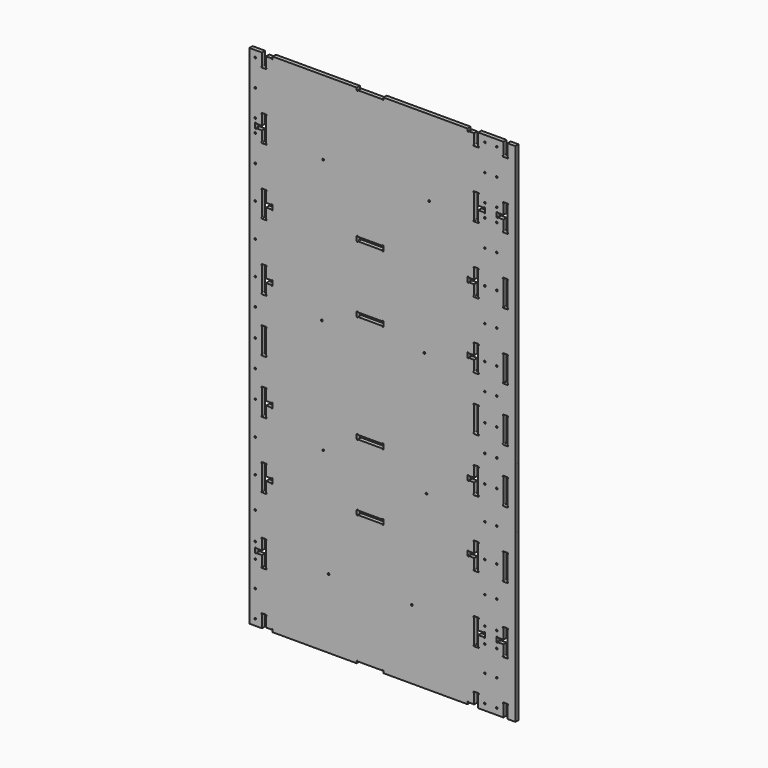
from build123d import *

# Parameters (mm, degrees)
F1_DEPTH = 18


# Not quite as in the source:
# - ends of sketch curves that miss each other by under 0.0002 mm in the source are joined


with BuildPart() as f1:
    # F0 (on Front) → F1 (new body)
    with BuildSketch(Plane.XZ):
        with BuildLine():
            Line((-600, 1199.999468), (-600, -1086.136016))
            Line((-600, -1086.136016), (-543.499769, -1086.136016))
            Line((-543.499769, -1086.136016), (-543.499943, -1032.405806))
            Line((-543.499943, -1032.405806), (-543.499943, -1032.174617))
            Line((-543.499943, -1032.174617), (-543.730427, -1032.15657))
            ThreePointArc((-543.730427, -1032.15657), (-546.5078390374, -1029.0353698433), (-543.4997759989, -1026.1358066805))
            Line((-543.4997759989, -1026.1358066805), (-524.999754, -1026.135811))
            ThreePointArc((-524.999754, -1026.135811), (-521.9825983148, -1029.0348123172), (-524.7687069622, -1032.1565165026))
            Line((-524.7687069622, -1032.1565165026), (-524.99995, -1032.173915))
            Line((-524.99995, -1032.173915), (-524.99995, -1032.405811))
            Line((-524.99995, -1032.405811), (-524.999963, -1077.135343))
            Line((-524.999963, -1077.135343), (-501.269768, -1077.135372))
            Line((-501.269768, -1077.135372), (-501.03858, -1077.135372))
            Line((-501.03858, -1077.135372), (-501.020531, -1076.904889))
            ThreePointArc((-501.020531, -1076.904889), (-497.8993183355, -1074.1274914801), (-494.9997686603, -1077.135567001))
            Line((-494.9997686603, -1077.135567001), (-494.999768, -1086.13591))
            Line((-494.999768, -1086.13591), (-115.999169, -1086.135994))
            Line((-115.999169, -1086.135994), (-115.999158, -1077.135038))
            ThreePointArc((-115.999158, -1077.135038), (-113.1001576807, -1074.1178813531), (-109.9784525722, -1076.9039889678))
            Line((-109.9784525722, -1076.9039889678), (-109.961054, -1077.135232))
            Line((-109.961054, -1077.135232), (-109.729158, -1077.135232))
            Line((-109.729158, -1077.135232), (-1.769047, -1077.135238))
            Line((-1.769047, -1077.135238), (-1.537858, -1077.135238))
            Line((-1.537858, -1077.135238), (-1.51981, -1076.904754))
            ThreePointArc((-1.51981, -1076.904754), (1.6014001334, -1074.1273523449), (4.5009533351, -1077.1354249995))
            Line((4.5009533351, -1077.1354249995), (4.50095, -1086.136029))
            Line((4.50095, -1086.136029), (383.501336, -1086.136077))
            Line((383.501336, -1086.136077), (383.501336, -1077.135157))
            ThreePointArc((383.501336, -1077.135157), (386.4003373172, -1074.1180013148), (389.5220415026, -1076.9041099622))
            Line((389.5220415026, -1076.9041099622), (389.53944, -1077.135353))
            Line((389.53944, -1077.135353), (389.771336, -1077.135353))
            Line((389.771336, -1077.135353), (413.501359, -1077.13536))
            Line((413.501359, -1077.13536), (413.500838, -1032.409536))
            Line((413.500838, -1032.409536), (413.500835, -1032.178347))
            Line((413.500835, -1032.178347), (413.270352, -1032.160302))
            ThreePointArc((413.270352, -1032.160302), (410.4929139851, -1029.0391253645), (413.5009520011, -1026.1395367213))
            Line((413.5009520011, -1026.1395367213), (432.000964, -1026.139536))
            ThreePointArc((432.000964, -1026.139536), (435.0181206469, -1029.0385363193), (432.2320130322, -1032.1602414278))
            Line((432.2320130322, -1032.1602414278), (432.00077, -1032.17764))
            Line((432.00077, -1032.17764), (432.00077, -1032.409536))
            Line((432.00077, -1032.409536), (432.00077, -1086.136231))
            Line((432.00077, -1086.136231), (545.500906, -1086.136191))
            Line((545.500906, -1086.136191), (545.5009, -1032.409575))
            Line((545.5009, -1032.409575), (545.5009, -1032.178387))
            Line((545.5009, -1032.178387), (545.270417, -1032.160338))
            ThreePointArc((545.270417, -1032.160338), (542.4930153257, -1029.0391283663), (545.5010869995, -1026.1395746665))
            Line((545.5010869995, -1026.1395746665), (564.001096, -1026.139575))
            ThreePointArc((564.001096, -1026.139575), (567.0182526469, -1029.0385753193), (564.2321450322, -1032.1602804278))
            Line((564.2321450322, -1032.1602804278), (564.000902, -1032.177679))
            Line((564.000902, -1032.177679), (564.000902, -1032.409575))
            Line((564.000902, -1032.409575), (564.000902, -1086.13627))
            Line((564.000902, -1086.13627), (599.501161, -1086.136207))
            Line((599.501161, -1086.136207), (599.476525, -336.389715))
            Line((599.476525, -336.389715), (599.501387, -336.281022))
            Line((599.501387, -336.281022), (599.476798, -64.752505))
            Line((599.476798, -64.752505), (599.501477, -64.644176))
            Line((599.501477, -64.644176), (599.50151, 1199.999468))
            Line((599.50151, 1199.999468), (564.0008530006, 1199.999468))
            Line((564.0008530006, 1199.999468), (564.000885, 1146.273847))
            Line((564.000885, 1146.273847), (564.000886, 1146.042659))
            Line((564.000886, 1146.042659), (564.231369, 1146.024611))
            ThreePointArc((564.231369, 1146.024611), (567.0087737308, 1142.9034028231), (564.0007020005, 1140.003846668))
            Line((564.0007020005, 1140.003846668), (545.501107, 1140.003831))
            ThreePointArc((545.501107, 1140.003831), (542.4839494495, 1142.9028288263), (545.2700529849, 1146.0245352004))
            Line((545.2700529849, 1146.0245352004), (545.501295, 1146.041935))
            Line((545.501295, 1146.041935), (545.501295, 1146.273831))
            Line((545.501295, 1146.273831), (545.5012470009, 1199.999468))
            Line((545.5012470009, 1199.999468), (432.0011330008, 1199.999468))
            Line((432.0011330008, 1199.999468), (432.001181, 1146.273729))
            Line((432.001181, 1146.273729), (432.001181, 1146.042541))
            Line((432.001181, 1146.042541), (432.231665, 1146.024492))
            ThreePointArc((432.231665, 1146.024492), (435.0090697698, 1142.9032848599), (432.0010000005, 1140.0037286696))
            Line((432.0010000005, 1140.0037286696), (413.500972, 1140.003713))
            ThreePointArc((413.500972, 1140.003713), (410.4838471243, 1142.902745364), (413.2699870123, 1146.0244198369))
            Line((413.2699870123, 1146.0244198369), (413.50123, 1146.041817))
            Line((413.50123, 1146.041817), (413.501232, 1146.273713))
            Line((413.501232, 1146.273713), (413.501705, 1190.999532))
            Line((413.501705, 1190.999532), (389.771678, 1190.999511))
            Line((389.771678, 1190.999511), (389.540489, 1190.999511))
            Line((389.540489, 1190.999511), (389.522441, 1190.769028))
            ThreePointArc((389.522441, 1190.769028), (386.4012338599, 1187.9916232302), (383.5016776696, 1190.9996929995))
            Line((383.5016776696, 1190.9996929995), (383.5016700007, 1199.999468))
            Line((383.5016700007, 1199.999468), (4.5012910004, 1199.999468))
            Line((4.5012910004, 1199.999468), (4.501299, 1190.998973))
            ThreePointArc((4.501299, 1190.998973), (1.6023016734, 1187.9818144687), (-1.5194052004, 1190.7679179849))
            Line((-1.5194052004, 1190.7679179849), (-1.536805, 1190.999161))
            Line((-1.536805, 1190.999161), (-1.768701, 1190.999161))
            Line((-1.768701, 1190.999161), (-109.728821, 1190.999064))
            Line((-109.728821, 1190.999064), (-109.96001, 1190.999064))
            Line((-109.96001, 1190.999064), (-109.978058, 1190.768581))
            ThreePointArc((-109.978058, 1190.768581), (-113.0992651401, 1187.9911762302), (-115.9988213304, 1190.9992459995))
            Line((-115.9988213304, 1190.9992459995), (-115.9988289997, 1199.999468))
            Line((-115.9988289997, 1199.999468), (-494.999817, 1199.999468))
            Line((-494.999817, 1199.999468), (-494.999811, 1190.998816))
            ThreePointArc((-494.999811, 1190.998816), (-497.8988058318, 1187.9816545637), (-501.0205159787, 1190.7677560016))
            Line((-501.0205159787, 1190.7677560016), (-501.037915, 1190.998999))
            Line((-501.037915, 1190.998999), (-501.269812, 1190.998998))
            Line((-501.269812, 1190.998998), (-524.999617, 1190.998955))
            Line((-524.999617, 1190.998955), (-524.999577, 1146.269424))
            Line((-524.999577, 1146.269424), (-524.999577, 1146.038235))
            Line((-524.999577, 1146.038235), (-524.769094, 1146.020187))
            ThreePointArc((-524.769094, 1146.020187), (-521.9916892302, 1142.8989798599), (-524.9997589995, 1139.9994236696))
            Line((-524.9997589995, 1139.9994236696), (-543.499783, 1139.999407))
            ThreePointArc((-543.499783, 1139.999407), (-546.5169415512, 1142.8984048254), (-543.7308370153, 1146.0201122032))
            Line((-543.7308370153, 1146.0201122032), (-543.499595, 1146.037511))
            Line((-543.499595, 1146.037511), (-543.499595, 1146.269407))
            Line((-543.499595, 1146.269407), (-543.499643, 1199.999468))
            Line((-543.499643, 1199.999468), (-600, 1199.999468))
        make_face()
        with BuildLine():
            ThreePointArc((-573.470016, -1054.269081), (-570.8183655706, -1055.3674305706), (-569.720016, -1058.019081))
            ThreePointArc((-569.720016, -1058.019081), (-570.8183655706, -1060.6707314294), (-573.470016, -1061.769081))
            ThreePointArc((-573.470016, -1061.769081), (-576.1216664294, -1060.6707314294), (-577.220016, -1058.019081))
            ThreePointArc((-577.220016, -1058.019081), (-576.1216664294, -1055.3674305706), (-573.470016, -1054.269081))
        make_face(mode=Mode.SUBTRACT)
        with BuildLine():
            ThreePointArc((-573.470016, -934.104401), (-570.8183655706, -935.2027505706), (-569.720016, -937.854401))
            ThreePointArc((-569.720016, -937.854401), (-570.8183655706, -940.5060514294), (-573.470016, -941.604401))
            ThreePointArc((-573.470016, -941.604401), (-576.1216664294, -940.5060514294), (-577.220016, -937.854401))
            ThreePointArc((-577.220016, -937.854401), (-576.1216664294, -935.2027505706), (-573.470016, -934.104401))
        make_face(mode=Mode.SUBTRACT)
        with BuildLine():
            ThreePointArc((-573.470016, -817.646713), (-570.8183655706, -818.7450625706), (-569.720016, -821.396713))
            ThreePointArc((-569.720016, -821.396713), (-570.8183655706, -824.0483634294), (-573.470016, -825.146713))
            ThreePointArc((-573.470016, -825.146713), (-576.1216664294, -824.0483634294), (-577.220016, -821.396713))
            ThreePointArc((-577.220016, -821.396713), (-576.1216664294, -818.7450625706), (-573.470016, -817.646713))
        make_face(mode=Mode.SUBTRACT)
        with BuildLine():
            ThreePointArc((-573.470016, -747.138491), (-570.8183655706, -748.2368405706), (-569.720016, -750.888491))
            ThreePointArc((-569.720016, -750.888491), (-570.8183655706, -753.5401414294), (-573.470016, -754.638491))
            ThreePointArc((-573.470016, -754.638491), (-576.1216664294, -753.5401414294), (-577.220016, -750.888491))
            ThreePointArc((-577.220016, -750.888491), (-576.1216664294, -748.2368405706), (-573.470016, -747.138491))
        make_face(mode=Mode.SUBTRACT)
        with BuildLine():
            Line((-568.483106, -777.131339), (-543.503058, -777.131347))
            Line((-543.503058, -777.131347), (-543.49994, -732.155506))
            ThreePointArc((-543.49994, -732.1555059928), (-546.5097319928, -729.1452975), (-543.499523, -726.1355060073))
            Line((-543.499523, -726.135506), (-524.999526, -726.135511))
            ThreePointArc((-524.999526, -726.135511), (-521.989527, -729.145512), (-524.999528, -732.155511))
            Line((-524.999528, -732.155511), (-524.99956, -840.615631))
            ThreePointArc((-524.99956, -840.615631), (-521.989561, -843.625632), (-524.999562, -846.635631))
            Line((-524.999562, -846.635631), (-543.499559, -846.635626))
            ThreePointArc((-543.499559, -846.6356259929), (-546.5097659929, -843.6258325), (-543.499972, -840.615626007))
            Line((-543.499972, -840.615626), (-543.503063, -795.631365))
            Line((-543.503063, -795.631365), (-568.483112, -795.631357))
            ThreePointArc((-568.483112, -795.631357), (-571.4931125, -798.641357), (-574.503112, -795.631356))
            Line((-574.503112, -795.631356), (-574.503106, -777.131338))
            ThreePointArc((-574.503106, -777.131338), (-571.4931055, -774.121339), (-568.483106, -777.131339))
        make_face(mode=Mode.SUBTRACT)
        with BuildLine():
            ThreePointArc((-573.470016, -622.138491), (-570.8183655706, -623.2368405706), (-569.720016, -625.888491))
            ThreePointArc((-569.720016, -625.888491), (-570.8183655706, -628.5401414294), (-573.470016, -629.638491))
            ThreePointArc((-573.470016, -629.638491), (-576.1216664294, -628.5401414294), (-577.220016, -625.888491))
            ThreePointArc((-577.220016, -625.888491), (-576.1216664294, -623.2368405706), (-573.470016, -622.138491))
        make_face(mode=Mode.SUBTRACT)
        with BuildLine():
            ThreePointArc((-239.337181, -773.063468), (-240.4635018729, -775.7826471271), (-243.182681, -776.908968))
            ThreePointArc((-243.182681, -776.908968), (-245.9018601271, -775.7826471271), (-247.028181, -773.063468))
            ThreePointArc((-247.028181, -773.063468), (-245.9018601271, -770.3442888729), (-243.182681, -769.217968))
            ThreePointArc((-243.182681, -769.217968), (-240.4635018729, -770.3442888729), (-239.337181, -773.063468))
        make_face(mode=Mode.SUBTRACT)
        with BuildLine():
            ThreePointArc((-573.470016, -482.494274), (-570.8183655706, -483.5926235706), (-569.720016, -486.244274))
            ThreePointArc((-569.720016, -486.244274), (-570.8183655706, -488.8959244294), (-573.470016, -489.994274))
            ThreePointArc((-573.470016, -489.994274), (-576.1216664294, -488.8959244294), (-577.220016, -486.244274))
            ThreePointArc((-577.220016, -486.244274), (-576.1216664294, -483.5926235706), (-573.470016, -482.494274))
        make_face(mode=Mode.SUBTRACT)
        with BuildLine():
            ThreePointArc((-543.499435, -546.634817), (-546.509434, -543.6248165), (-543.499434, -540.614817))
            Line((-543.499434, -540.614817), (-543.499401, -432.154696))
            ThreePointArc((-543.499401, -432.154696), (-546.5094, -429.144695), (-543.499399, -426.134696))
            Line((-543.499399, -426.134696), (-524.999523, -426.134709))
            ThreePointArc((-524.999523, -426.134709), (-521.989524, -429.1447095), (-524.999524, -432.154709))
            Line((-524.999524, -432.154709), (-524.999532, -477.135051))
            Line((-524.999532, -477.135051), (-501.018807, -477.135055))
            ThreePointArc((-501.018807, -477.135055), (-498.008806, -474.125056), (-494.998807, -477.135057))
            Line((-494.998807, -477.135057), (-494.998819, -495.634923))
            ThreePointArc((-494.998819, -495.634923), (-498.00882, -498.644922), (-501.018819, -495.634921))
            Line((-501.018819, -495.634921), (-524.999038, -495.634914))
            Line((-524.999038, -495.634914), (-524.999044, -540.614822))
            ThreePointArc((-524.999044, -540.614822), (-521.989044, -543.624822), (-524.999044, -546.634822))
            Line((-524.999044, -546.634822), (-543.499435, -546.634817))
        make_face(mode=Mode.SUBTRACT)
        with BuildLine():
            ThreePointArc((-573.470016, -332.494274), (-570.8183655706, -333.5926235706), (-569.720016, -336.244274))
            ThreePointArc((-569.720016, -336.244274), (-570.8183655706, -338.8959244294), (-573.470016, -339.994274))
            ThreePointArc((-573.470016, -339.994274), (-576.1216664294, -338.8959244294), (-577.220016, -336.244274))
            ThreePointArc((-577.220016, -336.244274), (-576.1216664294, -333.5926235706), (-573.470016, -332.494274))
        make_face(mode=Mode.SUBTRACT)
        with BuildLine():
            ThreePointArc((-573.470016, -182.494274), (-570.8183655706, -183.5926235706), (-569.720016, -186.244274))
            ThreePointArc((-569.720016, -186.244274), (-570.8183655706, -188.8959244294), (-573.470016, -189.994274))
            ThreePointArc((-573.470016, -189.994274), (-576.1216664294, -188.8959244294), (-577.220016, -186.244274))
            ThreePointArc((-577.220016, -186.244274), (-576.1216664294, -183.5926235706), (-573.470016, -182.494274))
        make_face(mode=Mode.SUBTRACT)
        with BuildLine():
            ThreePointArc((-543.499486, -246.6309949334), (-546.5101189334, -243.621628), (-543.500752, -240.6109950666))
            Line((-543.500752, -240.6109950666), (-543.523568, -132.150751))
            ThreePointArc((-543.523568, -132.150751), (-546.5342009334, -129.141384), (-543.524834, -126.1307510666))
            Line((-543.524834, -126.1307510666), (-525.024512, -126.139097))
            ThreePointArc((-525.024512, -126.139097), (-522.0130223688, -129.1476069999), (-525.0215319997, -132.1590966312))
            Line((-525.0215319997, -132.1590966312), (-524.999265, -177.134783))
            Line((-524.999265, -177.134783), (-501.044184, -177.138104))
            ThreePointArc((-501.044184, -177.138104), (-498.0337665, -174.128522029), (-495.0241840289, -177.138939))
            Line((-495.0241840289, -177.138939), (-495.024184, -195.634784))
            ThreePointArc((-495.024184, -195.634784), (-498.034185, -198.644783), (-501.044184, -195.634782))
            Line((-501.044184, -195.634782), (-524.999148, -195.634776))
            Line((-524.999148, -195.634776), (-524.999475, -240.611))
            ThreePointArc((-524.999475, -240.611), (-521.989497, -243.6210215), (-524.999518, -246.631))
            Line((-524.999518, -246.631), (-525.27493, -246.631))
            Line((-525.27493, -246.631), (-543.499486, -246.6309949334))
        make_face(mode=Mode.SUBTRACT)
        with BuildLine():
            ThreePointArc((-573.470016, -61.029942), (-570.8183655706, -62.1282915706), (-569.720016, -64.779942))
            ThreePointArc((-569.720016, -64.779942), (-570.8183655706, -67.4315924294), (-573.470016, -68.529942))
            ThreePointArc((-573.470016, -68.529942), (-576.1216664294, -67.4315924294), (-577.220016, -64.779942))
            ThreePointArc((-577.220016, -64.779942), (-576.1216664294, -62.1282915706), (-573.470016, -61.029942))
        make_face(mode=Mode.SUBTRACT)
        with BuildLine():
            ThreePointArc((4.501686, -495.635075), (1.491685, -498.645074), (-1.518314, -495.635073))
            Line((-1.518314, -495.635073), (-109.978434, -495.635041))
            ThreePointArc((-109.978434, -495.635041), (-112.988435, -498.64504), (-115.998434, -495.635039))
            Line((-115.998434, -495.635039), (-115.998429, -477.135021))
            ThreePointArc((-115.998429, -477.135021), (-112.988428, -474.125022), (-109.978429, -477.135023))
            Line((-109.978429, -477.135023), (-1.518309, -477.135055))
            ThreePointArc((-1.518309, -477.135055), (1.491692, -474.125056), (4.501691, -477.135057))
            Line((4.501691, -477.135057), (4.501686, -495.635075))
        make_face(mode=Mode.SUBTRACT)
        with BuildLine():
            ThreePointArc((-263.373181, -289.357468), (-264.4995018729, -292.0766471271), (-267.218681, -293.202968))
            ThreePointArc((-267.218681, -293.202968), (-269.9378601271, -292.0766471271), (-271.064181, -289.357468))
            ThreePointArc((-271.064181, -289.357468), (-269.9378601271, -286.6382888729), (-267.218681, -285.511968))
            ThreePointArc((-267.218681, -285.511968), (-264.4995018729, -286.6382888729), (-263.373181, -289.357468))
        make_face(mode=Mode.SUBTRACT)
        with BuildLine():
            ThreePointArc((-109.9783950019, -195.634943), (-112.9885035, -198.644834998), (-115.998394998, -195.634726))
            Line((-115.998395, -195.634726), (-116.024154, -177.134743))
            ThreePointArc((-116.0241539981, -177.134743), (-113.0140465, -174.1248510019), (-110.0041540019, -177.134958))
            Line((-110.004154, -177.134958), (-1.544028, -177.138844))
            ThreePointArc((-1.5440279981, -177.138844), (1.46608, -174.1289520019), (4.4759719981, -177.13906))
            Line((4.475972, -177.13906), (4.501737, -195.639079))
            ThreePointArc((4.501736998, -195.639079), (1.491628, -198.648969998), (-1.518262998, -195.638861))
            Line((-1.518263, -195.638861), (-109.978395, -195.634943))
        make_face(mode=Mode.SUBTRACT)
        with BuildLine():
            ThreePointArc((136.210819, -773.063468), (135.0844981271, -775.7826471271), (132.365319, -776.908968))
            ThreePointArc((132.365319, -776.908968), (129.6461398729, -775.7826471271), (128.519819, -773.063468))
            ThreePointArc((128.519819, -773.063468), (129.6461398729, -770.3442888729), (132.365319, -769.217968))
            ThreePointArc((132.365319, -769.217968), (135.0844981271, -770.3442888729), (136.210819, -773.063468))
        make_face(mode=Mode.SUBTRACT)
        with BuildLine():
            ThreePointArc((461.992812, -1054.269081), (464.6444624294, -1055.3674305706), (465.742812, -1058.019081))
            ThreePointArc((465.742812, -1058.019081), (464.6444624294, -1060.6707314294), (461.992812, -1061.769081))
            ThreePointArc((461.992812, -1061.769081), (459.3411615706, -1060.6707314294), (458.242812, -1058.019081))
            ThreePointArc((458.242812, -1058.019081), (459.3411615706, -1055.3674305706), (461.992812, -1054.269081))
        make_face(mode=Mode.SUBTRACT)
        with BuildLine():
            ThreePointArc((515.501476, -1054.269081), (518.1531264294, -1055.3674305706), (519.251476, -1058.019081))
            ThreePointArc((519.251476, -1058.019081), (518.1531264294, -1060.6707314294), (515.501476, -1061.769081))
            ThreePointArc((515.501476, -1061.769081), (512.8498255706, -1060.6707314294), (511.751476, -1058.019081))
            ThreePointArc((511.751476, -1058.019081), (512.8498255706, -1055.3674305706), (515.501476, -1054.269081))
        make_face(mode=Mode.SUBTRACT)
        with BuildLine():
            ThreePointArc((461.992812, -934.104401), (464.6444624294, -935.2027505706), (465.742812, -937.854401))
            ThreePointArc((465.742812, -937.854401), (464.6444624294, -940.5060514294), (461.992812, -941.604401))
            ThreePointArc((461.992812, -941.604401), (459.3411615706, -940.5060514294), (458.242812, -937.854401))
            ThreePointArc((458.242812, -937.854401), (459.3411615706, -935.2027505706), (461.992812, -934.104401))
        make_face(mode=Mode.SUBTRACT)
        with BuildLine():
            ThreePointArc((515.501476, -934.104401), (518.1531264294, -935.2027505706), (519.251476, -937.854401))
            ThreePointArc((519.251476, -937.854401), (518.1531264294, -940.5060514294), (515.501476, -941.604401))
            ThreePointArc((515.501476, -941.604401), (512.8498255706, -940.5060514294), (511.751476, -937.854401))
            ThreePointArc((511.751476, -937.854401), (512.8498255706, -935.2027505706), (515.501476, -934.104401))
        make_face(mode=Mode.SUBTRACT)
        with BuildLine():
            Line((456.978759, -795.631663), (431.99874, -795.631656))
            Line((431.99874, -795.631656), (432.000914, -840.61473))
            ThreePointArc((432.000914, -840.6147300035), (435.0110589965, -843.6245845), (432.001205, -846.6347299965))
            Line((432.001205, -846.63473), (413.501174, -846.634725))
            ThreePointArc((413.501174, -846.634725), (410.491175, -843.624724), (413.501176, -840.614725))
            Line((413.501176, -840.614725), (413.501209, -732.154554))
            ThreePointArc((413.501209, -732.154554), (410.491209, -729.1445535), (413.50121, -726.134554))
            Line((413.50121, -726.134554), (432.001241, -726.134559))
            ThreePointArc((432.001241, -726.1345590036), (435.0110939964, -729.1447065), (432.000946, -732.1545589964))
            Line((432.000946, -732.154559), (431.998749, -777.131638))
            Line((431.998749, -777.131638), (456.978764, -777.131645))
            ThreePointArc((456.978764, -777.131645), (459.988765, -774.121646), (462.998764, -777.131647))
            Line((462.998764, -777.131647), (462.998759, -795.631665))
            ThreePointArc((462.998759, -795.631665), (459.988758, -798.641664), (456.978759, -795.631663))
        make_face(mode=Mode.SUBTRACT)
        with BuildLine():
            ThreePointArc((461.992812, -817.646713), (464.6444624294, -818.7450625706), (465.742812, -821.396713))
            ThreePointArc((465.742812, -821.396713), (464.6444624294, -824.0483634294), (461.992812, -825.146713))
            ThreePointArc((461.992812, -825.146713), (459.3411615706, -824.0483634294), (458.242812, -821.396713))
            ThreePointArc((458.242812, -821.396713), (459.3411615706, -818.7450625706), (461.992812, -817.646713))
        make_face(mode=Mode.SUBTRACT)
        with BuildLine():
            ThreePointArc((461.992812, -747.138491), (464.6444624294, -748.2368405706), (465.742812, -750.888491))
            ThreePointArc((465.742812, -750.888491), (464.6444624294, -753.5401414294), (461.992812, -754.638491))
            ThreePointArc((461.992812, -754.638491), (459.3411615706, -753.5401414294), (458.242812, -750.888491))
            ThreePointArc((458.242812, -750.888491), (459.3411615706, -748.2368405706), (461.992812, -747.138491))
        make_face(mode=Mode.SUBTRACT)
        with BuildLine():
            ThreePointArc((515.501476, -817.646713), (518.1531264294, -818.7450625706), (519.251476, -821.396713))
            ThreePointArc((519.251476, -821.396713), (518.1531264294, -824.0483634294), (515.501476, -825.146713))
            ThreePointArc((515.501476, -825.146713), (512.8498255706, -824.0483634294), (511.751476, -821.396713))
            ThreePointArc((511.751476, -821.396713), (512.8498255706, -818.7450625706), (515.501476, -817.646713))
        make_face(mode=Mode.SUBTRACT)
        with BuildLine():
            ThreePointArc((515.501476, -747.138491), (518.1531264294, -748.2368405706), (519.251476, -750.888491))
            ThreePointArc((519.251476, -750.888491), (518.1531264294, -753.5401414294), (515.501476, -754.638491))
            ThreePointArc((515.501476, -754.638491), (512.8498255706, -753.5401414294), (511.751476, -750.888491))
            ThreePointArc((511.751476, -750.888491), (512.8498255706, -748.2368405706), (515.501476, -747.138491))
        make_face(mode=Mode.SUBTRACT)
        with BuildLine():
            ThreePointArc((520.516044, -795.631681), (517.506043, -798.64168), (514.496044, -795.631679))
            Line((514.496044, -795.631679), (514.49605, -777.131661))
            ThreePointArc((514.49605, -777.131661), (517.506051, -774.121662), (520.51605, -777.131663))
            Line((520.51605, -777.131663), (545.496097, -777.13167))
            Line((545.496097, -777.13167), (545.499022, -732.152738))
            ThreePointArc((545.499022, -732.1527379936), (542.4892180063, -729.1425425), (545.499413, -726.1327380063))
            Line((545.499413, -726.132738), (563.999415, -726.132744))
            ThreePointArc((563.999415, -726.132744), (567.009414, -729.142745), (563.999413, -732.152744))
            Line((563.999413, -732.152744), (563.999381, -840.612864))
            ThreePointArc((563.999381, -840.612864), (567.00938, -843.622865), (563.999379, -846.632864))
            Line((563.999379, -846.632864), (545.499378, -846.632858))
            ThreePointArc((545.499378, -846.6328579937), (542.4891840063, -843.623052), (545.49899, -840.6128580063))
            Line((545.49899, -840.612858), (545.496091, -795.631688))
            Line((545.496091, -795.631688), (520.516044, -795.631681))
        make_face(mode=Mode.SUBTRACT)
        with BuildLine():
            ThreePointArc((461.992812, -622.138491), (464.6444624294, -623.2368405706), (465.742812, -625.888491))
            ThreePointArc((465.742812, -625.888491), (464.6444624294, -628.5401414294), (461.992812, -629.638491))
            ThreePointArc((461.992812, -629.638491), (459.3411615706, -628.5401414294), (458.242812, -625.888491))
            ThreePointArc((458.242812, -625.888491), (459.3411615706, -623.2368405706), (461.992812, -622.138491))
        make_face(mode=Mode.SUBTRACT)
        with BuildLine():
            ThreePointArc((515.501476, -622.138491), (518.1531264294, -623.2368405706), (519.251476, -625.888491))
            ThreePointArc((519.251476, -625.888491), (518.1531264294, -628.5401414294), (515.501476, -629.638491))
            ThreePointArc((515.501476, -629.638491), (512.8498255706, -628.5401414294), (511.751476, -625.888491))
            ThreePointArc((511.751476, -625.888491), (512.8498255706, -623.2368405706), (515.501476, -622.138491))
        make_face(mode=Mode.SUBTRACT)
        with BuildLine():
            ThreePointArc((202.306819, -310.388468), (201.1804981271, -313.1076471271), (198.461319, -314.233968))
            ThreePointArc((198.461319, -314.233968), (195.7421398729, -313.1076471271), (194.615819, -310.388468))
            ThreePointArc((194.615819, -310.388468), (195.7421398729, -307.6692888729), (198.461319, -306.542968))
            ThreePointArc((198.461319, -306.542968), (201.1804981271, -307.6692888729), (202.306819, -310.388468))
        make_face(mode=Mode.SUBTRACT)
        with BuildLine():
            ThreePointArc((389.522068, -495.635077), (386.5120675, -498.645076), (383.502068, -495.635076))
            Line((383.502068, -495.635076), (383.502074, -477.135049))
            ThreePointArc((383.502074, -477.135049), (386.5120745, -474.125049), (389.522074, -477.13505))
            Line((389.522074, -477.13505), (413.502094, -477.135058))
            Line((413.502094, -477.135058), (413.501329, -432.154659))
            ThreePointArc((413.501329, -432.1546589996), (410.4912780004, -429.14471), (413.501227, -426.1346590004))
            Line((413.501227, -426.134659), (432.001249, -426.134665))
            ThreePointArc((432.001249, -426.134665), (435.011248, -429.144666), (432.001247, -432.154665))
            Line((432.001247, -432.154665), (432.001215, -540.614785))
            ThreePointArc((432.001215, -540.614785), (435.011214, -543.624786), (432.001213, -546.634785))
            Line((432.001213, -546.634785), (413.501191, -546.634779))
            ThreePointArc((413.501191, -546.6347789995), (410.4912440005, -543.624726), (413.501297, -540.6147790005))
            Line((413.501297, -540.614779), (413.502088, -495.635085))
            Line((413.502088, -495.635085), (389.522068, -495.635077))
        make_face(mode=Mode.SUBTRACT)
        with BuildLine():
            ThreePointArc((461.992812, -482.494274), (464.6444624294, -483.5926235706), (465.742812, -486.244274))
            ThreePointArc((465.742812, -486.244274), (464.6444624294, -488.8959244294), (461.992812, -489.994274))
            ThreePointArc((461.992812, -489.994274), (459.3411615706, -488.8959244294), (458.242812, -486.244274))
            ThreePointArc((458.242812, -486.244274), (459.3411615706, -483.5926235706), (461.992812, -482.494274))
        make_face(mode=Mode.SUBTRACT)
        with BuildLine():
            ThreePointArc((515.501476, -482.494274), (518.1531264294, -483.5926235706), (519.251476, -486.244274))
            ThreePointArc((519.251476, -486.244274), (518.1531264294, -488.8959244294), (515.501476, -489.994274))
            ThreePointArc((515.501476, -489.994274), (512.8498255706, -488.8959244294), (511.751476, -486.244274))
            ThreePointArc((511.751476, -486.244274), (512.8498255706, -483.5926235706), (515.501476, -482.494274))
        make_face(mode=Mode.SUBTRACT)
        with BuildLine():
            ThreePointArc((564.001479, -426.134706), (567.011478, -429.144707), (564.001477, -432.154706))
            Line((564.001477, -432.154706), (564.001445, -540.614826))
            ThreePointArc((564.001445, -540.614826), (567.011444, -543.624827), (564.001443, -546.634826))
            Line((564.001443, -546.634826), (545.501439, -546.63482))
            ThreePointArc((545.501439, -546.63482), (542.49144, -543.624819), (545.501441, -540.61482))
            Line((545.501441, -540.61482), (545.501473, -432.1547))
            ThreePointArc((545.501473, -432.1547), (542.491474, -429.144699), (545.501475, -426.1347))
            Line((545.501475, -426.1347), (564.001479, -426.134706))
        make_face(mode=Mode.SUBTRACT)
        with BuildLine():
            ThreePointArc((461.992812, -332.494274), (464.6444624294, -333.5926235706), (465.742812, -336.244274))
            ThreePointArc((465.742812, -336.244274), (464.6444624294, -338.8959244294), (461.992812, -339.994274))
            ThreePointArc((461.992812, -339.994274), (459.3411615706, -338.8959244294), (458.242812, -336.244274))
            ThreePointArc((458.242812, -336.244274), (459.3411615706, -333.5926235706), (461.992812, -332.494274))
        make_face(mode=Mode.SUBTRACT)
        with BuildLine():
            ThreePointArc((515.501476, -332.494274), (518.1531264294, -333.5926235706), (519.251476, -336.244274))
            ThreePointArc((519.251476, -336.244274), (518.1531264294, -338.8959244294), (515.501476, -339.994274))
            ThreePointArc((515.501476, -339.994274), (512.8498255706, -338.8959244294), (511.751476, -336.244274))
            ThreePointArc((511.751476, -336.244274), (512.8498255706, -333.5926235706), (515.501476, -332.494274))
        make_face(mode=Mode.SUBTRACT)
        with BuildLine():
            Line((413.498425, -240.614709), (413.476838, -195.639275))
            Line((413.476838, -195.639275), (389.521758, -195.635648))
            ThreePointArc((389.521758, -195.635648), (386.5113025, -198.6451919655), (383.5017580344, -195.634737))
            Line((383.5017580344, -195.634737), (383.501764, -177.139277))
            ThreePointArc((383.501764, -177.139277), (386.511765, -174.129278), (389.521764, -177.139279))
            Line((389.521764, -177.139279), (413.501667, -177.139286))
            Line((413.501667, -177.139286), (413.478779, -132.154528))
            ThreePointArc((413.478779, -132.154528), (410.4672473896, -129.1460595001), (413.4757159997, -126.1345283894))
            Line((413.4757159997, -126.1345283894), (431.975811, -126.139664))
            ThreePointArc((431.975811, -126.139664), (434.9864469328, -129.149028), (431.977083, -132.1596639328))
            Line((431.977083, -132.1596639328), (431.999995, -240.61979))
            ThreePointArc((431.999995, -240.61979), (435.0106309328, -243.629154), (432.001267, -246.6397899328))
            Line((432.001267, -246.6397899328), (413.501315, -246.634708))
            ThreePointArc((413.501315, -246.634708), (410.4898703468, -243.6261530001), (413.498425, -240.614709))
        make_face(mode=Mode.SUBTRACT)
        with BuildLine():
            ThreePointArc((461.992812, -182.494274), (464.6444624294, -183.5926235706), (465.742812, -186.244274))
            ThreePointArc((465.742812, -186.244274), (464.6444624294, -188.8959244294), (461.992812, -189.994274))
            ThreePointArc((461.992812, -189.994274), (459.3411615706, -188.8959244294), (458.242812, -186.244274))
            ThreePointArc((458.242812, -186.244274), (459.3411615706, -183.5926235706), (461.992812, -182.494274))
        make_face(mode=Mode.SUBTRACT)
        with BuildLine():
            ThreePointArc((515.501476, -182.494274), (518.1531264294, -183.5926235706), (519.251476, -186.244274))
            ThreePointArc((519.251476, -186.244274), (518.1531264294, -188.8959244294), (515.501476, -189.994274))
            ThreePointArc((515.501476, -189.994274), (512.8498255706, -188.8959244294), (511.751476, -186.244274))
            ThreePointArc((511.751476, -186.244274), (512.8498255706, -183.5926235706), (515.501476, -182.494274))
        make_face(mode=Mode.SUBTRACT)
        with BuildLine():
            ThreePointArc((563.976055, -126.1396340668), (566.9866889331, -129.1489995), (563.977324, -132.159633933))
            Line((563.977324, -132.159634), (564.000179, -240.619829))
            ThreePointArc((564.000179, -240.6198290668), (567.0108129332, -243.629195), (564.001447, -246.6398289332))
            Line((564.001447, -246.639829), (545.501352, -246.634752))
            ThreePointArc((545.501352, -246.634752), (542.491352, -243.6247515), (545.501353, -240.614752))
            Line((545.501353, -240.614752), (545.501386, -132.159628))
            ThreePointArc((545.501386, -132.159628), (542.491387, -129.149627), (545.501388, -126.139628))
            Line((545.501388, -126.139628), (563.976055, -126.139634))
        make_face(mode=Mode.SUBTRACT)
        with BuildLine():
            ThreePointArc((461.992812, -61.029942), (464.6444624294, -62.1282915706), (465.742812, -64.779942))
            ThreePointArc((465.742812, -64.779942), (464.6444624294, -67.4315924294), (461.992812, -68.529942))
            ThreePointArc((461.992812, -68.529942), (459.3411615706, -67.4315924294), (458.242812, -64.779942))
            ThreePointArc((458.242812, -64.779942), (459.3411615706, -62.1282915706), (461.992812, -61.029942))
        make_face(mode=Mode.SUBTRACT)
        with BuildLine():
            ThreePointArc((515.501476, -61.029942), (518.1531264294, -62.1282915706), (519.251476, -64.779942))
            ThreePointArc((519.251476, -64.779942), (518.1531264294, -67.4315924294), (515.501476, -68.529942))
            ThreePointArc((515.501476, -68.529942), (512.8498255706, -67.4315924294), (511.751476, -64.779942))
            ThreePointArc((511.751476, -64.779942), (512.8498255706, -62.1282915706), (515.501476, -61.029942))
        make_face(mode=Mode.SUBTRACT)
        with BuildLine():
            ThreePointArc((-573.470016, 60.663174), (-570.8183655706, 59.5648244294), (-569.720016, 56.913174))
            ThreePointArc((-569.720016, 56.913174), (-570.8183655706, 54.2615235706), (-573.470016, 53.163174))
            ThreePointArc((-573.470016, 53.163174), (-576.1216664294, 54.2615235706), (-577.220016, 56.913174))
            ThreePointArc((-577.220016, 56.913174), (-576.1216664294, 59.5648244294), (-573.470016, 60.663174))
        make_face(mode=Mode.SUBTRACT)
        with BuildLine():
            ThreePointArc((-543.499433, -3.319512), (-546.509433, -0.309512), (-543.499433, 2.700488))
            Line((-543.499433, 2.700488), (-543.499433, 111.160679))
            ThreePointArc((-543.499433, 111.160679), (-546.509433, 114.170679), (-543.499433, 117.180679))
            Line((-543.499433, 117.180679), (-524.999426, 117.180679))
            ThreePointArc((-524.999426, 117.180679), (-521.989426, 114.170679), (-524.999426, 111.160679))
            Line((-524.999426, 111.160679), (-524.999426, 2.700481))
            ThreePointArc((-524.999426, 2.700481), (-521.989426, -0.309519), (-524.999426, -3.319519))
            Line((-524.999426, -3.319519), (-543.499433, -3.319512))
        make_face(mode=Mode.SUBTRACT)
        with BuildLine():
            ThreePointArc((-573.470016, 184.428207), (-570.8183655706, 183.3298574294), (-569.720016, 180.678207))
            ThreePointArc((-569.720016, 180.678207), (-570.8183655706, 178.0265565706), (-573.470016, 176.928207))
            ThreePointArc((-573.470016, 176.928207), (-576.1216664294, 178.0265565706), (-577.220016, 180.678207))
            ThreePointArc((-577.220016, 180.678207), (-576.1216664294, 183.3298574294), (-573.470016, 184.428207))
        make_face(mode=Mode.SUBTRACT)
        with BuildLine():
            ThreePointArc((-573.470016, 303.975583), (-570.8183655706, 302.8772334294), (-569.720016, 300.225583))
            ThreePointArc((-569.720016, 300.225583), (-570.8183655706, 297.5739325706), (-573.470016, 296.475583))
            ThreePointArc((-573.470016, 296.475583), (-576.1216664294, 297.5739325706), (-577.220016, 300.225583))
            ThreePointArc((-577.220016, 300.225583), (-576.1216664294, 302.8772334294), (-573.470016, 303.975583))
        make_face(mode=Mode.SUBTRACT)
        with BuildLine():
            ThreePointArc((-543.499405, 239.995158), (-546.509406, 243.005157), (-543.499407, 246.015158))
            Line((-543.499407, 246.015158), (-543.49944, 354.475278))
            ThreePointArc((-543.49944, 354.475278), (-546.50944, 357.4852775), (-543.499441, 360.495278))
            Line((-543.499441, 360.495278), (-525.274932, 360.495284))
            Line((-525.274932, 360.495284), (-524.999425, 360.495284))
            ThreePointArc((-524.999425, 360.495284), (-521.989403, 357.485306), (-524.999381, 354.475284))
            Line((-524.999381, 354.475284), (-524.999054, 309.499058))
            Line((-524.999054, 309.499058), (-501.019028, 309.499065))
            ThreePointArc((-501.019028, 309.499065), (-498.009029, 312.509066), (-494.999028, 309.499067))
            Line((-494.999028, 309.499067), (-494.999022, 290.99904))
            ThreePointArc((-494.999022, 290.99904), (-498.009021, 287.989039), (-501.019022, 290.999038))
            Line((-501.019022, 290.999038), (-524.999049, 290.999031))
            Line((-524.999049, 290.999031), (-524.999349, 246.015164))
            ThreePointArc((-524.999349, 246.015164), (-521.989369, 243.005144), (-524.999389, 239.995164))
            Line((-524.999389, 239.995164), (-543.499405, 239.995158))
        make_face(mode=Mode.SUBTRACT)
        with BuildLine():
            ThreePointArc((-573.470016, 454.037237), (-570.8183655706, 452.9388874294), (-569.720016, 450.287237))
            ThreePointArc((-569.720016, 450.287237), (-570.8183655706, 447.6355865706), (-573.470016, 446.537237))
            ThreePointArc((-573.470016, 446.537237), (-576.1216664294, 447.6355865706), (-577.220016, 450.287237))
            ThreePointArc((-577.220016, 450.287237), (-576.1216664294, 452.9388874294), (-573.470016, 454.037237))
        make_face(mode=Mode.SUBTRACT)
        with BuildLine():
            ThreePointArc((-269.381181, 224.392532), (-270.5075018729, 221.6733528729), (-273.226681, 220.547032))
            ThreePointArc((-273.226681, 220.547032), (-275.9458601271, 221.6733528729), (-277.072181, 224.392532))
            ThreePointArc((-277.072181, 224.392532), (-275.9458601271, 227.1117111271), (-273.226681, 228.238032))
            ThreePointArc((-273.226681, 228.238032), (-270.5075018729, 227.1117111271), (-269.381181, 224.392532))
        make_face(mode=Mode.SUBTRACT)
        Polygon((-83.952804, 57.290199), (-66.39547, 57.290199), (-66.39547, 37.319532), (-83.952804, 37.319532), (-84.447179, 37.322936), (-84.938684, 37.351886), (-85.426384, 37.405993), (-85.909345, 37.484866), (-86.386635, 37.588113), (-86.857319, 37.715345), (-87.320465, 37.86617), (-87.775137, 38.040199), (-88.220403, 38.23704), (-88.65533, 38.456303), (-89.078983, 38.697597), (-89.490429, 38.960532), (-89.888734, 39.244717), (-90.272965, 39.549761), (-90.642189, 39.875274), (-90.99547, 40.220866), (-91.335909, 40.572373), (-91.656981, 40.939303), (-91.958318, 41.320764), (-92.239554, 41.715866), (-92.500321, 42.123717), (-92.740252, 42.543428), (-92.95898, 42.974108), (-93.156137, 43.414866), (-93.331357, 43.864811), (-93.484273, 44.323053), (-93.614516, 44.788702), (-93.72172, 45.260866), (-93.805519, 45.738655), (-93.865543, 46.221178), (-93.901427, 46.707545), (-93.912804, 47.196866), (-93.915773, 47.698427), (-93.892934, 48.19748), (-93.844665, 48.69308), (-93.771345, 49.184282), (-93.673354, 49.67014), (-93.551069, 50.149709), (-93.404871, 50.622044), (-93.235137, 51.086199), (-93.042247, 51.541229), (-92.82658, 51.986189), (-92.588514, 52.420133), (-92.328429, 52.842116), (-92.046703, 53.251192), (-91.743715, 53.646418), (-91.419845, 54.026846), (-91.07547, 54.391532), (-90.715343, 54.735658), (-90.339575, 55.059788), (-89.949088, 55.36355), (-89.544804, 55.646574), (-89.127645, 55.908489), (-88.698533, 56.148923), (-88.25839, 56.367506), (-87.808137, 56.563866), (-87.348697, 56.737632), (-86.880991, 56.888433), (-86.405942, 57.015899), (-85.92447, 57.119657), (-85.437499, 57.199338), (-84.94595, 57.254569), (-84.450744, 57.28498), align=None, mode=Mode.SUBTRACT)
        Polygon((-40.233259, 77.836764), (-39.81947, 77.839532), (-39.399604, 77.842936), (-38.980634, 77.835696), (-38.562752, 77.817889), (-38.146153, 77.78959), (-37.731028, 77.750875), (-37.31757, 77.701819), (-36.905973, 77.6425), (-36.496429, 77.572991), (-36.089131, 77.493368), (-35.684272, 77.403709), (-35.282045, 77.304087), (-34.882642, 77.194579), (-34.486257, 77.075261), (-34.093083, 76.946207), (-33.703312, 76.807495), (-33.317137, 76.659199), (-32.934751, 76.501395), (-32.556347, 76.334159), (-32.182118, 76.157567), (-31.812257, 75.971694), (-31.446956, 75.776616), (-31.086409, 75.572408), (-30.730807, 75.359147), (-30.380345, 75.136907), (-30.035215, 74.905766), (-29.69561, 74.665797), (-29.361723, 74.417078), (-29.033746, 74.159683), (-28.711873, 73.893689), (-28.396297, 73.619171), (-28.087209, 73.336205), (-27.784804, 73.044866), (-27.434944, 72.664584), (-27.095422, 72.276396), (-26.766329, 71.880535), (-26.447752, 71.477235), (-26.13978, 71.06673), (-25.842503, 70.649254), (-25.556009, 70.225041), (-25.280387, 69.794324), (-25.015726, 69.357338), (-24.762115, 68.914316), (-24.519642, 68.465492), (-24.288398, 68.0111), (-24.068469, 67.551374), (-23.859946, 67.086549), (-23.662917, 66.616857), (-23.47747, 66.142532), (-23.303696, 65.66381), (-23.141683, 65.180922), (-22.991519, 64.694104), (-22.853293, 64.20359), (-22.727095, 63.709612), (-22.613013, 63.212405), (-22.511137, 62.712204), (-22.421554, 62.209241), (-22.344354, 61.70375), (-22.279625, 61.195967), (-22.227458, 60.686123), (-22.187939, 60.174454), (-22.161159, 59.661193), (-22.147206, 59.146575), (-22.146169, 58.630832), (-22.158137, 58.114199), (-22.142066, 57.553078), (-22.140288, 56.992888), (-22.152705, 56.433889), (-22.17922, 55.87634), (-22.219735, 55.320499), (-22.274153, 54.766627), (-22.342375, 54.214982), (-22.424304, 53.665824), (-22.519842, 53.119412), (-22.628892, 52.576006), (-22.751357, 52.035864), (-22.887137, 51.499246), (-23.036136, 50.966411), (-23.198257, 50.437619), (-23.373401, 49.913128), (-23.56147, 49.393199), (-23.762368, 48.87809), (-23.975996, 48.36806), (-24.202258, 47.86337), (-24.441054, 47.364277), (-24.692288, 46.871042), (-24.955861, 46.383924), (-25.231677, 45.903181), (-25.519637, 45.429074), (-25.819644, 44.961861), (-26.131601, 44.501802), (-26.455409, 44.049157), (-26.79097, 43.604183), (-27.138189, 43.167142), (-27.496965, 42.738291), (-27.867203, 42.31789), (-28.248804, 41.906199), (-28.534552, 41.615525), (-28.827168, 41.333058), (-29.126454, 41.058878), (-29.432215, 40.793069), (-29.744256, 40.53571), (-30.06238, 40.286885), (-30.386392, 40.046673), (-30.716095, 39.815157), (-31.051295, 39.592419), (-31.391795, 39.378539), (-31.7374, 39.1736), (-32.087913, 38.977683), (-32.443139, 38.79087), (-32.802883, 38.613241), (-33.166947, 38.444879), (-33.535137, 38.285866), (-33.907257, 38.136282), (-34.28311, 37.996209), (-34.662502, 37.865729), (-35.045236, 37.744923), (-35.431117, 37.633873), (-35.819948, 37.532661), (-36.211534, 37.441367), (-36.605679, 37.360074), (-37.002187, 37.288863), (-37.400863, 37.227816), (-37.801511, 37.177013), (-38.203934, 37.136538), (-38.607937, 37.10647), (-39.013325, 37.086892), (-39.419902, 37.077886), (-39.82747, 37.079532), (-40.241719, 37.083206), (-40.654831, 37.09767), (-41.06661, 37.12284), (-41.476856, 37.158631), (-41.885372, 37.20496), (-42.291959, 37.261741), (-42.696419, 37.328891), (-43.098554, 37.406324), (-43.498165, 37.493956), (-43.895055, 37.591704), (-44.289025, 37.699481), (-44.679877, 37.817204), (-45.067412, 37.944789), (-45.451433, 38.08215), (-45.83174, 38.229204), (-46.208137, 38.385866), (-46.580424, 38.552051), (-46.948404, 38.727675), (-47.311878, 38.912653), (-47.670648, 39.106902), (-48.024515, 39.310336), (-48.373282, 39.522871), (-48.71675, 39.744423), (-49.05472, 39.974907), (-49.386996, 40.214239), (-49.713378, 40.462334), (-50.033668, 40.719107), (-50.347668, 40.984475), (-50.65518, 41.258353), (-50.956006, 41.540655), (-51.249946, 41.831299), (-51.536804, 42.130199), (-51.906984, 42.539727), (-52.265963, 42.957642), (-52.613649, 43.383691), (-52.94995, 43.817621), (-53.274774, 44.259177), (-53.58803, 44.708107), (-53.889626, 45.164157), (-54.17947, 45.627074), (-54.457471, 46.096604), (-54.723536, 46.572494), (-54.977573, 47.05449), (-55.219491, 47.54234), (-55.449199, 48.035789), (-55.666603, 48.534584), (-55.871613, 49.038472), (-56.064137, 49.547199), (-56.244083, 50.060512), (-56.411358, 50.578158), (-56.565872, 51.099883), (-56.707533, 51.625433), (-56.836248, 52.154556), (-56.951926, 52.686998), (-57.054475, 53.222505), (-57.143804, 53.760824), (-57.21982, 54.301702), (-57.282431, 54.844885), (-57.331547, 55.390119), (-57.367075, 55.937152), (-57.388923, 56.48573), (-57.396999, 57.035599), (-57.391212, 57.586507), (-57.37147, 58.138199), (-57.3799, 58.653027), (-57.375249, 59.166852), (-57.35761, 59.679438), (-57.327075, 60.190548), (-57.283734, 60.699945), (-57.227681, 61.207392), (-57.159007, 61.712653), (-57.077804, 62.215491), (-56.984163, 62.715668), (-56.878176, 63.212948), (-56.759936, 63.707095), (-56.629533, 64.197871), (-56.48706, 64.685039), (-56.332608, 65.168364), (-56.16627, 65.647607), (-55.988137, 66.122532), (-55.798301, 66.592903), (-55.596853, 67.058482), (-55.383886, 67.519033), (-55.159491, 67.974319), (-54.92376, 68.424103), (-54.676786, 68.868148), (-54.418658, 69.306217), (-54.14947, 69.738074), (-53.869314, 70.163482), (-53.57828, 70.582204), (-53.276462, 70.994002), (-52.96395, 71.398642), (-52.640836, 71.795884), (-52.307213, 72.185494), (-51.963171, 72.567233), (-51.608804, 72.940866), (-51.314898, 73.232079), (-51.014304, 73.515167), (-50.707212, 73.790051), (-50.393809, 74.056652), (-50.074283, 74.314892), (-49.748821, 74.564692), (-49.417613, 74.805973), (-49.080845, 75.038657), (-48.738707, 75.262666), (-48.391385, 75.47792), (-48.039068, 75.684341), (-47.681944, 75.88185), (-47.320201, 76.070369), (-46.954027, 76.249819), (-46.58361, 76.420122), (-46.209137, 76.581199), (-45.830797, 76.732971), (-45.448778, 76.87536), (-45.063268, 77.008287), (-44.674455, 77.131673), (-44.282526, 77.24544), (-43.88767, 77.34951), (-43.490075, 77.443803), (-43.089929, 77.528241), (-42.687419, 77.602745), (-42.282734, 77.667237), (-41.876062, 77.721639), (-41.46759, 77.765871), (-41.057507, 77.799855), (-40.646001, 77.823512), align=None, mode=Mode.SUBTRACT)
        with BuildLine():
            ThreePointArc((-115.998649, 309.499022), (-112.98865, 312.509023), (-109.978649, 309.499024))
            Line((-109.978649, 309.499024), (-1.518523, 309.499056))
            ThreePointArc((-1.518523, 309.499056), (1.491476, 312.509057), (4.501477, 309.499058))
            Line((4.501477, 309.499058), (4.501482, 290.999076))
            ThreePointArc((4.501482, 290.999076), (1.491483, 287.989075), (-1.518518, 290.999074))
            Line((-1.518518, 290.999074), (-109.978643, 290.999042))
            ThreePointArc((-109.978643, 290.999042), (-112.988642, 287.989041), (-115.998643, 290.99904))
            Line((-115.998643, 290.99904), (-115.998649, 309.499022))
        make_face(mode=Mode.SUBTRACT)
        with BuildLine():
            ThreePointArc((-573.470016, 604.037237), (-570.8183655706, 602.9388874294), (-569.720016, 600.287237))
            ThreePointArc((-569.720016, 600.287237), (-570.8183655706, 597.6355865706), (-573.470016, 596.537237))
            ThreePointArc((-573.470016, 596.537237), (-576.1216664294, 597.6355865706), (-577.220016, 600.287237))
            ThreePointArc((-577.220016, 600.287237), (-576.1216664294, 602.9388874294), (-573.470016, 604.037237))
        make_face(mode=Mode.SUBTRACT)
        with BuildLine():
            ThreePointArc((-543.499311, 539.998984), (-546.509312, 543.008983), (-543.499313, 546.018984))
            Line((-543.499313, 546.018984), (-543.499345, 654.479104))
            ThreePointArc((-543.499345, 654.479104), (-546.509346, 657.489103), (-543.499347, 660.499104))
            Line((-543.499347, 660.499104), (-524.998956, 660.499109))
            ThreePointArc((-524.998956, 660.499109), (-521.988955, 657.48911), (-524.998954, 654.479109))
            Line((-524.998954, 654.479109), (-524.998941, 609.499198))
            Line((-524.998941, 609.499198), (-501.018721, 609.499205))
            ThreePointArc((-501.018721, 609.499205), (-498.008722, 612.509206), (-494.998721, 609.499207))
            Line((-494.998721, 609.499207), (-494.99871, 590.99934))
            ThreePointArc((-494.99871, 590.99934), (-498.0087095, 587.98934), (-501.01871, 590.999339))
            Line((-501.01871, 590.999339), (-524.999435, 590.999335))
            Line((-524.999435, 590.999335), (-524.999427, 546.018993))
            ThreePointArc((-524.999427, 546.018993), (-521.989427, 543.0089935), (-524.999426, 539.998993))
            Line((-524.999426, 539.998993), (-543.499311, 539.998984))
        make_face(mode=Mode.SUBTRACT)
        with BuildLine():
            ThreePointArc((-573.470016, 754.037237), (-570.8183655706, 752.9388874294), (-569.720016, 750.287237))
            ThreePointArc((-569.720016, 750.287237), (-570.8183655706, 747.6355865706), (-573.470016, 746.537237))
            ThreePointArc((-573.470016, 746.537237), (-576.1216664294, 747.6355865706), (-577.220016, 750.287237))
            ThreePointArc((-577.220016, 750.287237), (-576.1216664294, 752.9388874294), (-573.470016, 754.037237))
        make_face(mode=Mode.SUBTRACT)
        with BuildLine():
            ThreePointArc((-573.470016, 874.037237), (-570.8183655706, 872.9388874294), (-569.720016, 870.287237))
            ThreePointArc((-569.720016, 870.287237), (-570.8183655706, 867.6355865706), (-573.470016, 866.537237))
            ThreePointArc((-573.470016, 866.537237), (-576.1216664294, 867.6355865706), (-577.220016, 870.287237))
            ThreePointArc((-577.220016, 870.287237), (-576.1216664294, 872.9388874294), (-573.470016, 874.037237))
        make_face(mode=Mode.SUBTRACT)
        with BuildLine():
            ThreePointArc((-573.470016, 934.037237), (-570.8183655706, 932.9388874294), (-569.720016, 930.287237))
            ThreePointArc((-569.720016, 930.287237), (-570.8183655706, 927.6355865706), (-573.470016, 926.537237))
            ThreePointArc((-573.470016, 926.537237), (-576.1216664294, 927.6355865706), (-577.220016, 930.287237))
            ThreePointArc((-577.220016, 930.287237), (-576.1216664294, 932.9388874294), (-573.470016, 934.037237))
        make_face(mode=Mode.SUBTRACT)
        with BuildLine():
            Line((-543.499846, 846.019789), (-543.502961, 890.99563))
            Line((-543.502961, 890.99563), (-568.483009, 890.995623))
            ThreePointArc((-568.483009, 890.995623), (-571.493008, 887.985622), (-574.503009, 890.995621))
            Line((-574.503009, 890.995621), (-574.503014, 909.495639))
            ThreePointArc((-574.503014, 909.495639), (-571.493015, 912.50564), (-568.483014, 909.495641))
            Line((-568.483014, 909.495641), (-543.502966, 909.495648))
            Line((-543.502966, 909.495648), (-543.499879, 954.479909))
            ThreePointArc((-543.499879, 954.4799090071), (-546.5096719929, 957.490116), (-543.499465, 960.4999089929))
            Line((-543.499465, 960.499909), (-524.999465, 960.499915))
            ThreePointArc((-524.999465, 960.499915), (-521.989464, 957.489916), (-524.999463, 954.479915))
            Line((-524.999463, 954.479915), (-524.99943, 846.019795))
            ThreePointArc((-524.99943, 846.019795), (-521.98943, 843.0097955), (-524.999429, 839.999795))
            Line((-524.999429, 839.999795), (-543.499429, 839.999789))
            ThreePointArc((-543.499429, 839.9997890073), (-546.5096379928, 843.0095805), (-543.499846, 846.0197889928))
        make_face(mode=Mode.SUBTRACT)
        with BuildLine():
            ThreePointArc((-573.470016, 1054.037237), (-570.8183655706, 1052.9388874294), (-569.720016, 1050.287237))
            ThreePointArc((-569.720016, 1050.287237), (-570.8183655706, 1047.6355865706), (-573.470016, 1046.537237))
            ThreePointArc((-573.470016, 1046.537237), (-576.1216664294, 1047.6355865706), (-577.220016, 1050.287237))
            ThreePointArc((-577.220016, 1050.287237), (-576.1216664294, 1052.9388874294), (-573.470016, 1054.037237))
        make_face(mode=Mode.SUBTRACT)
        with BuildLine():
            ThreePointArc((-573.470016, 1174.217247), (-570.8183655706, 1173.1188974294), (-569.720016, 1170.467247))
            ThreePointArc((-569.720016, 1170.467247), (-570.8183655706, 1167.8155965706), (-573.470016, 1166.717247))
            ThreePointArc((-573.470016, 1166.717247), (-576.1216664294, 1167.8155965706), (-577.220016, 1170.467247))
            ThreePointArc((-577.220016, 1170.467247), (-576.1216664294, 1173.1188974294), (-573.470016, 1174.217247))
        make_face(mode=Mode.SUBTRACT)
        with BuildLine():
            ThreePointArc((-263.373181, 864.326532), (-264.4995018729, 861.6073528729), (-267.218681, 860.481032))
            ThreePointArc((-267.218681, 860.481032), (-269.9378601271, 861.6073528729), (-271.064181, 864.326532))
            ThreePointArc((-271.064181, 864.326532), (-269.9378601271, 867.0457111271), (-267.218681, 868.172032))
            ThreePointArc((-267.218681, 868.172032), (-264.4995018729, 867.0457111271), (-263.373181, 864.326532))
        make_face(mode=Mode.SUBTRACT)
        with BuildLine():
            ThreePointArc((4.501789, 590.99934), (1.49179, 587.989339), (-1.518211, 590.999338))
            Line((-1.518211, 590.999338), (-109.978331, 590.999306))
            ThreePointArc((-109.978331, 590.999306), (-112.98833, 587.989305), (-115.998331, 590.999304))
            Line((-115.998331, 590.999304), (-115.998337, 609.499322))
            ThreePointArc((-115.998337, 609.499322), (-112.988338, 612.509323), (-109.978337, 609.499324))
            Line((-109.978337, 609.499324), (-1.518217, 609.499356))
            ThreePointArc((-1.518217, 609.499356), (1.491782, 612.509357), (4.501783, 609.499358))
            Line((4.501783, 609.499358), (4.501789, 590.99934))
        make_face(mode=Mode.SUBTRACT)
        Polygon((4.012074, 77.836764), (4.425863, 77.839532), (4.845729, 77.842936), (5.264699, 77.835696), (5.682581, 77.817889), (6.099181, 77.78959), (6.514306, 77.750875), (6.927763, 77.701819), (7.339361, 77.6425), (7.748905, 77.572991), (8.156202, 77.493368), (8.561061, 77.403709), (8.963289, 77.304087), (9.362691, 77.194579), (9.759076, 77.075261), (10.15225, 76.946207), (10.542021, 76.807495), (10.928196, 76.659199), (11.310582, 76.501395), (11.688986, 76.334159), (12.063215, 76.157567), (12.433076, 75.971694), (12.798377, 75.776616), (13.158925, 75.572408), (13.514526, 75.359147), (13.864988, 75.136907), (14.210118, 74.905766), (14.549723, 74.665797), (14.88361, 74.417078), (15.211587, 74.159683), (15.53346, 73.893689), (15.849037, 73.619171), (16.158124, 73.336205), (16.46053, 73.044866), (16.81039, 72.664584), (17.149911, 72.276396), (17.479005, 71.880535), (17.797582, 71.477235), (18.105553, 71.06673), (18.40283, 70.649254), (18.689324, 70.225041), (18.964946, 69.794324), (19.229607, 69.357338), (19.483218, 68.914316), (19.725691, 68.465492), (19.956936, 68.0111), (20.176864, 67.551374), (20.385388, 67.086549), (20.582417, 66.616857), (20.767863, 66.142532), (20.941637, 65.66381), (21.103651, 65.180922), (21.253815, 64.694104), (21.39204, 64.20359), (21.518238, 63.709612), (21.63232, 63.212405), (21.734197, 62.712204), (21.82378, 62.209241), (21.90098, 61.70375), (21.965708, 61.195967), (22.017876, 60.686123), (22.057394, 60.174454), (22.084174, 59.661193), (22.098127, 59.146575), (22.099164, 58.630832), (22.087196, 58.114199), (22.103267, 57.553078), (22.105045, 56.992888), (22.092628, 56.433889), (22.066113, 55.87634), (22.025598, 55.320499), (21.971181, 54.766627), (21.902959, 54.214982), (21.82103, 53.665824), (21.725491, 53.119412), (21.616441, 52.576006), (21.493977, 52.035864), (21.358196, 51.499246), (21.209197, 50.966411), (21.047076, 50.437619), (20.871933, 49.913128), (20.683863, 49.393199), (20.482965, 48.87809), (20.269337, 48.36806), (20.043076, 47.86337), (19.80428, 47.364277), (19.553046, 46.871042), (19.289472, 46.383924), (19.013657, 45.903181), (18.725696, 45.429074), (18.425689, 44.961861), (18.113733, 44.501802), (17.789925, 44.049157), (17.454363, 43.604183), (17.107145, 43.167142), (16.748368, 42.738291), (16.37813, 42.31789), (15.99653, 41.906199), (15.710781, 41.615525), (15.418166, 41.333058), (15.118879, 41.058878), (14.813118, 40.793069), (14.501077, 40.53571), (14.182953, 40.286885), (13.858942, 40.046673), (13.529238, 39.815157), (13.194038, 39.592419), (12.853538, 39.378539), (12.507933, 39.1736), (12.15742, 38.977683), (11.802194, 38.79087), (11.442451, 38.613241), (11.078386, 38.444879), (10.710196, 38.285866), (10.338077, 38.136282), (9.962223, 37.996209), (9.582831, 37.865729), (9.200097, 37.744923), (8.814217, 37.633873), (8.425386, 37.532661), (8.0338, 37.441367), (7.639655, 37.360074), (7.243146, 37.288863), (6.84447, 37.227816), (6.443823, 37.177013), (6.041399, 37.136538), (5.637396, 37.10647), (5.232008, 37.086892), (4.825432, 37.077886), (4.417863, 37.079532), (4.003615, 37.083206), (3.590502, 37.09767), (3.178724, 37.12284), (2.768477, 37.158631), (2.359962, 37.20496), (1.953375, 37.261741), (1.548914, 37.328891), (1.14678, 37.406324), (0.747168, 37.493956), (0.350278, 37.591704), (-0.043692, 37.699481), (-0.434543, 37.817204), (-0.822079, 37.944789), (-1.206099, 38.08215), (-1.586407, 38.229204), (-1.962804, 38.385866), (-2.335091, 38.552051), (-2.703071, 38.727675), (-3.066545, 38.912653), (-3.425314, 39.106902), (-3.779182, 39.310336), (-4.127948, 39.522871), (-4.471416, 39.744423), (-4.809387, 39.974907), (-5.141663, 40.214239), (-5.468045, 40.462334), (-5.788335, 40.719107), (-6.102335, 40.984475), (-6.409847, 41.258353), (-6.710672, 41.540655), (-7.004613, 41.831299), (-7.29147, 42.130199), (-7.66165, 42.539727), (-8.020629, 42.957642), (-8.368315, 43.383691), (-8.704616, 43.817621), (-9.029441, 44.259177), (-9.342697, 44.708107), (-9.644293, 45.164157), (-9.934137, 45.627074), (-10.212137, 46.096604), (-10.478202, 46.572494), (-10.73224, 47.05449), (-10.974158, 47.54234), (-11.203865, 48.035789), (-11.42127, 48.534584), (-11.62628, 49.038472), (-11.818804, 49.547199), (-11.998749, 50.060512), (-12.166025, 50.578158), (-12.320539, 51.099883), (-12.4622, 51.625433), (-12.590915, 52.154556), (-12.706593, 52.686998), (-12.809142, 53.222505), (-12.89847, 53.760824), (-12.974486, 54.301702), (-13.037098, 54.844885), (-13.086214, 55.390119), (-13.121741, 55.937152), (-13.143589, 56.48573), (-13.151666, 57.035599), (-13.145879, 57.586507), (-13.126137, 58.138199), (-13.134566, 58.653027), (-13.129916, 59.166852), (-13.112277, 59.679438), (-13.081741, 60.190548), (-13.038401, 60.699945), (-12.982348, 61.207392), (-12.913674, 61.712653), (-12.83247, 62.215491), (-12.738829, 62.715668), (-12.632843, 63.212948), (-12.514602, 63.707095), (-12.3842, 64.197871), (-12.241727, 64.685039), (-12.087275, 65.168364), (-11.920937, 65.647607), (-11.742804, 66.122532), (-11.552968, 66.592903), (-11.35152, 67.058482), (-11.138553, 67.519033), (-10.914158, 67.974319), (-10.678427, 68.424103), (-10.431452, 68.868148), (-10.173325, 69.306217), (-9.904137, 69.738074), (-9.623981, 70.163482), (-9.332947, 70.582204), (-9.031128, 70.994002), (-8.718616, 71.398642), (-8.395503, 71.795884), (-8.061879, 72.185494), (-7.717838, 72.567233), (-7.36347, 72.940866), (-7.069564, 73.232079), (-6.768971, 73.515167), (-6.461879, 73.790051), (-6.148476, 74.056652), (-5.828949, 74.314892), (-5.503488, 74.564692), (-5.17228, 74.805973), (-4.835512, 75.038657), (-4.493374, 75.262666), (-4.146052, 75.47792), (-3.793735, 75.684341), (-3.436611, 75.88185), (-3.074868, 76.070369), (-2.708694, 76.249819), (-2.338276, 76.420122), (-1.963804, 76.581199), (-1.585464, 76.732971), (-1.203445, 76.87536), (-0.817935, 77.008287), (-0.429121, 77.131673), (-0.037193, 77.24544), (0.357663, 77.34951), (0.755258, 77.443803), (1.155405, 77.528241), (1.557914, 77.602745), (1.962599, 77.667237), (2.369271, 77.721639), (2.777743, 77.765871), (3.187826, 77.799855), (3.599332, 77.823512), align=None, mode=Mode.SUBTRACT)
        with BuildLine():
            ThreePointArc((193.293819, 245.423532), (192.1674981271, 242.7043528729), (189.448319, 241.578032))
            ThreePointArc((189.448319, 241.578032), (186.7291398729, 242.7043528729), (185.602819, 245.423532))
            ThreePointArc((185.602819, 245.423532), (186.7291398729, 248.1427111271), (189.448319, 249.269032))
            ThreePointArc((189.448319, 249.269032), (192.1674981271, 248.1427111271), (193.293819, 245.423532))
        make_face(mode=Mode.SUBTRACT)
        with BuildLine():
            ThreePointArc((432.001322, 117.178805), (435.011322, 114.168805), (432.001322, 111.158805))
            Line((432.001322, 111.158805), (432.001322, 2.698614))
            ThreePointArc((432.001322, 2.698614), (435.011322, -0.311386), (432.001322, -3.321386))
            Line((432.001322, -3.321386), (413.501316, -3.321393))
            ThreePointArc((413.501316, -3.321393), (410.491316, -0.311393), (413.501316, 2.698607))
            Line((413.501316, 2.698607), (413.501315, 111.158805))
            ThreePointArc((413.501315, 111.158805), (410.491315, 114.168805), (413.501315, 117.178805))
            Line((413.501315, 117.178805), (432.001322, 117.178805))
        make_face(mode=Mode.SUBTRACT)
        with BuildLine():
            ThreePointArc((461.992812, 60.663174), (464.6444624294, 59.5648244294), (465.742812, 56.913174))
            ThreePointArc((465.742812, 56.913174), (464.6444624294, 54.2615235706), (461.992812, 53.163174))
            ThreePointArc((461.992812, 53.163174), (459.3411615706, 54.2615235706), (458.242812, 56.913174))
            ThreePointArc((458.242812, 56.913174), (459.3411615706, 59.5648244294), (461.992812, 60.663174))
        make_face(mode=Mode.SUBTRACT)
        with BuildLine():
            ThreePointArc((515.501476, 60.663174), (518.1531264294, 59.5648244294), (519.251476, 56.913174))
            ThreePointArc((519.251476, 56.913174), (518.1531264294, 54.2615235706), (515.501476, 53.163174))
            ThreePointArc((515.501476, 53.163174), (512.8498255706, 54.2615235706), (511.751476, 56.913174))
            ThreePointArc((511.751476, 56.913174), (512.8498255706, 59.5648244294), (515.501476, 60.663174))
        make_face(mode=Mode.SUBTRACT)
        with BuildLine():
            ThreePointArc((545.501457, -3.319512), (542.491457, -0.309512), (545.501457, 2.700488))
            Line((545.501457, 2.700488), (545.501457, 111.160679))
            ThreePointArc((545.501457, 111.160679), (542.491457, 114.170679), (545.501457, 117.180679))
            Line((545.501457, 117.180679), (564.001464, 117.180679))
            ThreePointArc((564.001464, 117.180679), (567.011464, 114.170679), (564.001464, 111.160679))
            Line((564.001464, 111.160679), (564.001464, 2.700481))
            ThreePointArc((564.001464, 2.700481), (567.011464, -0.309519), (564.001464, -3.319519))
            Line((564.001464, -3.319519), (545.501457, -3.319512))
        make_face(mode=Mode.SUBTRACT)
        with BuildLine():
            ThreePointArc((461.992812, 184.428207), (464.6444624294, 183.3298574294), (465.742812, 180.678207))
            ThreePointArc((465.742812, 180.678207), (464.6444624294, 178.0265565706), (461.992812, 176.928207))
            ThreePointArc((461.992812, 176.928207), (459.3411615706, 178.0265565706), (458.242812, 180.678207))
            ThreePointArc((458.242812, 180.678207), (459.3411615706, 183.3298574294), (461.992812, 184.428207))
        make_face(mode=Mode.SUBTRACT)
        with BuildLine():
            ThreePointArc((515.501476, 184.428207), (518.1531264294, 183.3298574294), (519.251476, 180.678207))
            ThreePointArc((519.251476, 180.678207), (518.1531264294, 178.0265565706), (515.501476, 176.928207))
            ThreePointArc((515.501476, 176.928207), (512.8498255706, 178.0265565706), (511.751476, 180.678207))
            ThreePointArc((511.751476, 180.678207), (512.8498255706, 183.3298574294), (515.501476, 184.428207))
        make_face(mode=Mode.SUBTRACT)
        with BuildLine():
            Line((389.521856, 309.49906), (413.501878, 309.499067))
            Line((413.501878, 309.499067), (413.501381, 354.479064))
            ThreePointArc((413.501381, 354.4790640002), (410.4913480002, 357.4890305), (413.501314, 360.4990639998))
            Line((413.501314, 360.499064), (432.001335, 360.49907))
            ThreePointArc((432.001335, 360.49907), (435.011336, 357.489071), (432.001337, 354.47907))
            Line((432.001337, 354.47907), (432.001369, 246.018898))
            ThreePointArc((432.001369, 246.018898), (435.01137, 243.008899), (432.001371, 239.998898))
            Line((432.001371, 239.998898), (413.50135, 239.998893))
            ThreePointArc((413.50135, 239.9988930002), (410.4913810002, 243.0089245), (413.501413, 246.0188929998))
            Line((413.501413, 246.018893), (413.501883, 290.99904))
            Line((413.501883, 290.99904), (389.521861, 290.999033))
            ThreePointArc((389.521861, 290.999033), (386.511862, 287.989032), (383.501861, 290.999031))
            Line((383.501861, 290.999031), (383.501856, 309.499058))
            ThreePointArc((383.501856, 309.499058), (386.511855, 312.509059), (389.521856, 309.49906))
        make_face(mode=Mode.SUBTRACT)
        with BuildLine():
            ThreePointArc((461.992812, 303.975583), (464.6444624294, 302.8772334294), (465.742812, 300.225583))
            ThreePointArc((465.742812, 300.225583), (464.6444624294, 297.5739325706), (461.992812, 296.475583))
            ThreePointArc((461.992812, 296.475583), (459.3411615706, 297.5739325706), (458.242812, 300.225583))
            ThreePointArc((458.242812, 300.225583), (459.3411615706, 302.8772334294), (461.992812, 303.975583))
        make_face(mode=Mode.SUBTRACT)
        with BuildLine():
            ThreePointArc((515.501476, 303.975583), (518.1531264294, 302.8772334294), (519.251476, 300.225583))
            ThreePointArc((519.251476, 300.225583), (518.1531264294, 297.5739325706), (515.501476, 296.475583))
            ThreePointArc((515.501476, 296.475583), (512.8498255706, 297.5739325706), (511.751476, 300.225583))
            ThreePointArc((511.751476, 300.225583), (512.8498255706, 302.8772334294), (515.501476, 303.975583))
        make_face(mode=Mode.SUBTRACT)
        with BuildLine():
            ThreePointArc((564.001467, 360.499109), (567.011468, 357.48911), (564.001469, 354.479109))
            Line((564.001469, 354.479109), (564.001501, 246.01899))
            ThreePointArc((564.001501, 246.01899), (567.011502, 243.008991), (564.001503, 239.99899))
            Line((564.001503, 239.99899), (545.501485, 239.998931))
            ThreePointArc((545.501485, 239.998931), (542.491484, 243.00893), (545.501483, 246.018931))
            Line((545.501483, 246.018931), (545.501451, 354.479104))
            ThreePointArc((545.501451, 354.479104), (542.49145, 357.489103), (545.501449, 360.499104))
            Line((545.501449, 360.499104), (564.001467, 360.499109))
        make_face(mode=Mode.SUBTRACT)
        with BuildLine():
            ThreePointArc((461.992812, 454.037237), (464.6444624294, 452.9388874294), (465.742812, 450.287237))
            ThreePointArc((465.742812, 450.287237), (464.6444624294, 447.6355865706), (461.992812, 446.537237))
            ThreePointArc((461.992812, 446.537237), (459.3411615706, 447.6355865706), (458.242812, 450.287237))
            ThreePointArc((458.242812, 450.287237), (459.3411615706, 452.9388874294), (461.992812, 454.037237))
        make_face(mode=Mode.SUBTRACT)
        with BuildLine():
            ThreePointArc((515.501476, 454.037237), (518.1531264294, 452.9388874294), (519.251476, 450.287237))
            ThreePointArc((519.251476, 450.287237), (518.1531264294, 447.6355865706), (515.501476, 446.537237))
            ThreePointArc((515.501476, 446.537237), (512.8498255706, 447.6355865706), (511.751476, 450.287237))
            ThreePointArc((511.751476, 450.287237), (512.8498255706, 452.9388874294), (515.501476, 454.037237))
        make_face(mode=Mode.SUBTRACT)
        with BuildLine():
            ThreePointArc((214.324819, 855.313532), (213.1984981271, 852.5943528729), (210.479319, 851.468032))
            ThreePointArc((210.479319, 851.468032), (207.7601398729, 852.5943528729), (206.633819, 855.313532))
            ThreePointArc((206.633819, 855.313532), (207.7601398729, 858.0327111271), (210.479319, 859.159032))
            ThreePointArc((210.479319, 859.159032), (213.1984981271, 858.0327111271), (214.324819, 855.313532))
        make_face(mode=Mode.SUBTRACT)
        with BuildLine():
            Line((413.501414, 546.018944), (413.502188, 590.99934))
            Line((413.502188, 590.99934), (389.522168, 590.999333))
            ThreePointArc((389.522168, 590.999333), (386.512169, 587.989332), (383.502168, 590.999331))
            Line((383.502168, 590.999331), (383.502162, 609.499358))
            ThreePointArc((383.502162, 609.499358), (386.512161, 612.509359), (389.522162, 609.49936))
            Line((389.522162, 609.49936), (413.502182, 609.499367))
            Line((413.502182, 609.499367), (413.501382, 654.479064))
            ThreePointArc((413.501382, 654.4790640005), (410.4913280005, 657.48901), (413.501274, 660.4990639995))
            Line((413.501274, 660.499064), (432.001297, 660.49907))
            ThreePointArc((432.001297, 660.49907), (435.011298, 657.489071), (432.001299, 654.47907))
            Line((432.001299, 654.47907), (432.001331, 546.01895))
            ThreePointArc((432.001331, 546.01895), (435.011332, 543.008951), (432.001333, 539.99895))
            Line((432.001333, 539.99895), (413.50131, 539.998944))
            ThreePointArc((413.50131, 539.9989440004), (410.4913620004, 543.008996), (413.501414, 546.0189439996))
        make_face(mode=Mode.SUBTRACT)
        with BuildLine():
            ThreePointArc((461.992812, 604.037237), (464.6444624294, 602.9388874294), (465.742812, 600.287237))
            ThreePointArc((465.742812, 600.287237), (464.6444624294, 597.6355865706), (461.992812, 596.537237))
            ThreePointArc((461.992812, 596.537237), (459.3411615706, 597.6355865706), (458.242812, 600.287237))
            ThreePointArc((458.242812, 600.287237), (459.3411615706, 602.9388874294), (461.992812, 604.037237))
        make_face(mode=Mode.SUBTRACT)
        with BuildLine():
            ThreePointArc((515.501476, 604.037237), (518.1531264294, 602.9388874294), (519.251476, 600.287237))
            ThreePointArc((519.251476, 600.287237), (518.1531264294, 597.6355865706), (515.501476, 596.537237))
            ThreePointArc((515.501476, 596.537237), (512.8498255706, 597.6355865706), (511.751476, 600.287237))
            ThreePointArc((511.751476, 600.287237), (512.8498255706, 602.9388874294), (515.501476, 604.037237))
        make_face(mode=Mode.SUBTRACT)
        with BuildLine():
            ThreePointArc((564.00154, 660.499109), (567.011541, 657.48911), (564.001542, 654.479109))
            Line((564.001542, 654.479109), (564.001574, 546.018989))
            ThreePointArc((564.001574, 546.018989), (567.011575, 543.00899), (564.001576, 539.998989))
            Line((564.001576, 539.998989), (545.501558, 539.998984))
            ThreePointArc((545.501558, 539.998984), (542.491557, 543.008983), (545.501556, 546.018984))
            Line((545.501556, 546.018984), (545.501524, 654.479104))
            ThreePointArc((545.501524, 654.479104), (542.491523, 657.489103), (545.501522, 660.499104))
            Line((545.501522, 660.499104), (564.00154, 660.499109))
        make_face(mode=Mode.SUBTRACT)
        with BuildLine():
            ThreePointArc((461.992812, 754.037237), (464.6444624294, 752.9388874294), (465.742812, 750.287237))
            ThreePointArc((465.742812, 750.287237), (464.6444624294, 747.6355865706), (461.992812, 746.537237))
            ThreePointArc((461.992812, 746.537237), (459.3411615706, 747.6355865706), (458.242812, 750.287237))
            ThreePointArc((458.242812, 750.287237), (459.3411615706, 752.9388874294), (461.992812, 754.037237))
        make_face(mode=Mode.SUBTRACT)
        with BuildLine():
            ThreePointArc((515.501476, 754.037237), (518.1531264294, 752.9388874294), (519.251476, 750.287237))
            ThreePointArc((519.251476, 750.287237), (518.1531264294, 747.6355865706), (515.501476, 746.537237))
            ThreePointArc((515.501476, 746.537237), (512.8498255706, 747.6355865706), (511.751476, 750.287237))
            ThreePointArc((511.751476, 750.287237), (512.8498255706, 752.9388874294), (515.501476, 754.037237))
        make_face(mode=Mode.SUBTRACT)
        with BuildLine():
            ThreePointArc((461.992812, 874.037237), (464.6444624294, 872.9388874294), (465.742812, 870.287237))
            ThreePointArc((465.742812, 870.287237), (464.6444624294, 867.6355865706), (461.992812, 866.537237))
            ThreePointArc((461.992812, 866.537237), (459.3411615706, 867.6355865706), (458.242812, 870.287237))
            ThreePointArc((458.242812, 870.287237), (459.3411615706, 872.9388874294), (461.992812, 874.037237))
        make_face(mode=Mode.SUBTRACT)
        with BuildLine():
            ThreePointArc((515.501476, 874.037237), (518.1531264294, 872.9388874294), (519.251476, 870.287237))
            ThreePointArc((519.251476, 870.287237), (518.1531264294, 867.6355865706), (515.501476, 866.537237))
            ThreePointArc((515.501476, 866.537237), (512.8498255706, 867.6355865706), (511.751476, 870.287237))
            ThreePointArc((511.751476, 870.287237), (512.8498255706, 872.9388874294), (515.501476, 874.037237))
        make_face(mode=Mode.SUBTRACT)
        with BuildLine():
            ThreePointArc((432.001041, 846.0188469964), (435.0111879964, 843.008994), (432.001335, 839.9988470036))
            Line((432.001335, 839.998847), (413.501333, 839.998837))
            ThreePointArc((413.501333, 839.998837), (410.491332, 843.008836), (413.501331, 846.018837))
            Line((413.501331, 846.018837), (413.501298, 954.479008))
            ThreePointArc((413.501298, 954.479008), (410.491297, 957.4890075), (413.501297, 960.499008))
            Line((413.501297, 960.499008), (432.001299, 960.499014))
            ThreePointArc((432.001299, 960.4990139965), (435.0111539965, 957.488869), (432.001009, 954.4790140035))
            Line((432.001009, 954.479014), (431.998837, 909.495939))
            Line((431.998837, 909.495939), (456.978856, 909.495947))
            ThreePointArc((456.978856, 909.495947), (459.988855, 912.505948), (462.998856, 909.495949))
            Line((462.998856, 909.495949), (462.998861, 890.995931))
            ThreePointArc((462.998861, 890.995931), (459.988862, 887.98593), (456.978861, 890.995929))
            Line((456.978861, 890.995929), (431.998844, 890.995921))
            Line((431.998844, 890.995921), (432.001041, 846.018847))
        make_face(mode=Mode.SUBTRACT)
        with BuildLine():
            ThreePointArc((461.992812, 934.037237), (464.6444624294, 932.9388874294), (465.742812, 930.287237))
            ThreePointArc((465.742812, 930.287237), (464.6444624294, 927.6355865706), (461.992812, 926.537237))
            ThreePointArc((461.992812, 926.537237), (459.3411615706, 927.6355865706), (458.242812, 930.287237))
            ThreePointArc((458.242812, 930.287237), (459.3411615706, 932.9388874294), (461.992812, 934.037237))
        make_face(mode=Mode.SUBTRACT)
        with BuildLine():
            ThreePointArc((515.501476, 934.037237), (518.1531264294, 932.9388874294), (519.251476, 930.287237))
            ThreePointArc((519.251476, 930.287237), (518.1531264294, 927.6355865706), (515.501476, 926.537237))
            ThreePointArc((515.501476, 926.537237), (512.8498255706, 927.6355865706), (511.751476, 930.287237))
            ThreePointArc((511.751476, 930.287237), (512.8498255706, 932.9388874294), (515.501476, 934.037237))
        make_face(mode=Mode.SUBTRACT)
        with BuildLine():
            ThreePointArc((520.517882, 890.995948), (517.507883, 887.985947), (514.497882, 890.995946))
            Line((514.497882, 890.995946), (514.497876, 909.495964))
            ThreePointArc((514.497876, 909.495964), (517.507875, 912.505965), (520.517876, 909.495966))
            Line((520.517876, 909.495966), (545.497923, 909.495973))
            Line((545.497923, 909.495973), (545.500822, 954.477143))
            ThreePointArc((545.500822, 954.4771430063), (542.4910160062, 957.4873365), (545.501209, 960.4971429938))
            Line((545.501209, 960.497143), (564.001211, 960.497149))
            ThreePointArc((564.001211, 960.497149), (567.011212, 957.48715), (564.001213, 954.477149))
            Line((564.001213, 954.477149), (564.001245, 846.017029))
            ThreePointArc((564.001245, 846.017029), (567.011246, 843.00703), (564.001247, 839.997029))
            Line((564.001247, 839.997029), (545.501245, 839.997023))
            ThreePointArc((545.501245, 839.9970230063), (542.4910500063, 843.0068275), (545.500854, 846.0170229936))
            Line((545.500854, 846.017023), (545.497929, 890.995955))
            Line((545.497929, 890.995955), (520.517882, 890.995948))
        make_face(mode=Mode.SUBTRACT)
        with BuildLine():
            ThreePointArc((461.992812, 1054.037237), (464.6444624294, 1052.9388874294), (465.742812, 1050.287237))
            ThreePointArc((465.742812, 1050.287237), (464.6444624294, 1047.6355865706), (461.992812, 1046.537237))
            ThreePointArc((461.992812, 1046.537237), (459.3411615706, 1047.6355865706), (458.242812, 1050.287237))
            ThreePointArc((458.242812, 1050.287237), (459.3411615706, 1052.9388874294), (461.992812, 1054.037237))
        make_face(mode=Mode.SUBTRACT)
        with BuildLine():
            ThreePointArc((515.501476, 1054.037237), (518.1531264294, 1052.9388874294), (519.251476, 1050.287237))
            ThreePointArc((519.251476, 1050.287237), (518.1531264294, 1047.6355865706), (515.501476, 1046.537237))
            ThreePointArc((515.501476, 1046.537237), (512.8498255706, 1047.6355865706), (511.751476, 1050.287237))
            ThreePointArc((511.751476, 1050.287237), (512.8498255706, 1052.9388874294), (515.501476, 1054.037237))
        make_face(mode=Mode.SUBTRACT)
        with BuildLine():
            ThreePointArc((461.992812, 1174.217247), (464.6444624294, 1173.1188974294), (465.742812, 1170.467247))
            ThreePointArc((465.742812, 1170.467247), (464.6444624294, 1167.8155965706), (461.992812, 1166.717247))
            ThreePointArc((461.992812, 1166.717247), (459.3411615706, 1167.8155965706), (458.242812, 1170.467247))
            ThreePointArc((458.242812, 1170.467247), (459.3411615706, 1173.1188974294), (461.992812, 1174.217247))
        make_face(mode=Mode.SUBTRACT)
        with BuildLine():
            ThreePointArc((515.501476, 1174.217247), (518.1531264294, 1173.1188974294), (519.251476, 1170.467247))
            ThreePointArc((519.251476, 1170.467247), (518.1531264294, 1167.8155965706), (515.501476, 1166.717247))
            ThreePointArc((515.501476, 1166.717247), (512.8498255706, 1167.8155965706), (511.751476, 1170.467247))
            ThreePointArc((511.751476, 1170.467247), (512.8498255706, 1173.1188974294), (515.501476, 1174.217247))
        make_face(mode=Mode.SUBTRACT)
        Polygon((-66.39547, 37.319532), (-66.39547, 57.290199), (-83.952804, 57.290199), (-84.450744, 57.28498), (-84.94595, 57.254569), (-85.437499, 57.199338), (-85.92447, 57.119657), (-86.405942, 57.015899), (-86.880991, 56.888433), (-87.348697, 56.737632), (-87.808137, 56.563866), (-88.25839, 56.367506), (-88.698533, 56.148923), (-89.127645, 55.908489), (-89.544804, 55.646574), (-89.949088, 55.36355), (-90.339575, 55.059788), (-90.715343, 54.735658), (-91.07547, 54.391532), (-91.419845, 54.026846), (-91.743715, 53.646418), (-92.046703, 53.251192), (-92.328429, 52.842116), (-92.588514, 52.420133), (-92.82658, 51.986189), (-93.042247, 51.541229), (-93.235137, 51.086199), (-93.404871, 50.622044), (-93.551069, 50.149709), (-93.673354, 49.67014), (-93.771345, 49.184282), (-93.844665, 48.69308), (-93.892934, 48.19748), (-93.915773, 47.698427), (-93.912804, 47.196866), (-93.901427, 46.707545), (-93.865543, 46.221178), (-93.805519, 45.738655), (-93.72172, 45.260866), (-93.614516, 44.788702), (-93.484273, 44.323053), (-93.331357, 43.864811), (-93.156137, 43.414866), (-92.95898, 42.974108), (-92.740252, 42.543428), (-92.500321, 42.123717), (-92.239554, 41.715866), (-91.958318, 41.320764), (-91.656981, 40.939303), (-91.335909, 40.572373), (-90.99547, 40.220866), (-90.642189, 39.875274), (-90.272965, 39.549761), (-89.888734, 39.244717), (-89.490429, 38.960532), (-89.078983, 38.697597), (-88.65533, 38.456303), (-88.220403, 38.23704), (-87.775137, 38.040199), (-87.320465, 37.86617), (-86.857319, 37.715345), (-86.386635, 37.588113), (-85.909345, 37.484866), (-85.426384, 37.405993), (-84.938684, 37.351886), (-84.447179, 37.322936), (-83.952804, 37.319532), align=None)
        Polygon((-39.399604, 77.842936), (-39.81947, 77.839532), (-40.233259, 77.836764), (-40.646001, 77.823512), (-41.057507, 77.799855), (-41.46759, 77.765871), (-41.876062, 77.721639), (-42.282734, 77.667237), (-42.687419, 77.602745), (-43.089929, 77.528241), (-43.490075, 77.443803), (-43.88767, 77.34951), (-44.282526, 77.24544), (-44.674455, 77.131673), (-45.063268, 77.008287), (-45.448778, 76.87536), (-45.830797, 76.732971), (-46.209137, 76.581199), (-46.58361, 76.420122), (-46.954027, 76.249819), (-47.320201, 76.070369), (-47.681944, 75.88185), (-48.039068, 75.684341), (-48.391385, 75.47792), (-48.738707, 75.262666), (-49.080845, 75.038657), (-49.417613, 74.805973), (-49.748821, 74.564692), (-50.074283, 74.314892), (-50.393809, 74.056652), (-50.707212, 73.790051), (-51.014304, 73.515167), (-51.314898, 73.232079), (-51.608804, 72.940866), (-51.963171, 72.567233), (-52.307213, 72.185494), (-52.640836, 71.795884), (-52.96395, 71.398642), (-53.276462, 70.994002), (-53.57828, 70.582204), (-53.869314, 70.163482), (-54.14947, 69.738074), (-54.418658, 69.306217), (-54.676786, 68.868148), (-54.92376, 68.424103), (-55.159491, 67.974319), (-55.383886, 67.519033), (-55.596853, 67.058482), (-55.798301, 66.592903), (-55.988137, 66.122532), (-56.16627, 65.647607), (-56.332608, 65.168364), (-56.48706, 64.685039), (-56.629533, 64.197871), (-56.759936, 63.707095), (-56.878176, 63.212948), (-56.984163, 62.715668), (-57.077804, 62.215491), (-57.159007, 61.712653), (-57.227681, 61.207392), (-57.283734, 60.699945), (-57.327075, 60.190548), (-57.35761, 59.679438), (-57.375249, 59.166852), (-57.3799, 58.653027), (-57.37147, 58.138199), (-57.391212, 57.586507), (-57.396999, 57.035599), (-57.388923, 56.48573), (-57.367075, 55.937152), (-57.331547, 55.390119), (-57.282431, 54.844885), (-57.21982, 54.301702), (-57.143804, 53.760824), (-57.054475, 53.222505), (-56.951926, 52.686998), (-56.836248, 52.154556), (-56.707533, 51.625433), (-56.565872, 51.099883), (-56.411358, 50.578158), (-56.244083, 50.060512), (-56.064137, 49.547199), (-55.871613, 49.038472), (-55.666603, 48.534584), (-55.449199, 48.035789), (-55.219491, 47.54234), (-54.977573, 47.05449), (-54.723536, 46.572494), (-54.457471, 46.096604), (-54.17947, 45.627074), (-53.889626, 45.164157), (-53.58803, 44.708107), (-53.274774, 44.259177), (-52.94995, 43.817621), (-52.613649, 43.383691), (-52.265963, 42.957642), (-51.906984, 42.539727), (-51.536804, 42.130199), (-51.249946, 41.831299), (-50.956006, 41.540655), (-50.65518, 41.258353), (-50.347668, 40.984475), (-50.033668, 40.719107), (-49.713378, 40.462334), (-49.386996, 40.214239), (-49.05472, 39.974907), (-48.71675, 39.744423), (-48.373282, 39.522871), (-48.024515, 39.310336), (-47.670648, 39.106902), (-47.311878, 38.912653), (-46.948404, 38.727675), (-46.580424, 38.552051), (-46.208137, 38.385866), (-45.83174, 38.229204), (-45.451433, 38.08215), (-45.067412, 37.944789), (-44.679877, 37.817204), (-44.289025, 37.699481), (-43.895055, 37.591704), (-43.498165, 37.493956), (-43.098554, 37.406324), (-42.696419, 37.328891), (-42.291959, 37.261741), (-41.885372, 37.20496), (-41.476856, 37.158631), (-41.06661, 37.12284), (-40.654831, 37.09767), (-40.241719, 37.083206), (-39.82747, 37.079532), (-39.419902, 37.077886), (-39.013325, 37.086892), (-38.607937, 37.10647), (-38.203934, 37.136538), (-37.801511, 37.177013), (-37.400863, 37.227816), (-37.002187, 37.288863), (-36.605679, 37.360074), (-36.211534, 37.441367), (-35.819948, 37.532661), (-35.431117, 37.633873), (-35.045236, 37.744923), (-34.662502, 37.865729), (-34.28311, 37.996209), (-33.907257, 38.136282), (-33.535137, 38.285866), (-33.166947, 38.444879), (-32.802883, 38.613241), (-32.443139, 38.79087), (-32.087913, 38.977683), (-31.7374, 39.1736), (-31.391795, 39.378539), (-31.051295, 39.592419), (-30.716095, 39.815157), (-30.386392, 40.046673), (-30.06238, 40.286885), (-29.744256, 40.53571), (-29.432215, 40.793069), (-29.126454, 41.058878), (-28.827168, 41.333058), (-28.534552, 41.615525), (-28.248804, 41.906199), (-27.867203, 42.31789), (-27.496965, 42.738291), (-27.138189, 43.167142), (-26.79097, 43.604183), (-26.455409, 44.049157), (-26.131601, 44.501802), (-25.819644, 44.961861), (-25.519637, 45.429074), (-25.231677, 45.903181), (-24.955861, 46.383924), (-24.692288, 46.871042), (-24.441054, 47.364277), (-24.202258, 47.86337), (-23.975996, 48.36806), (-23.762368, 48.87809), (-23.56147, 49.393199), (-23.373401, 49.913128), (-23.198257, 50.437619), (-23.036136, 50.966411), (-22.887137, 51.499246), (-22.751357, 52.035864), (-22.628892, 52.576006), (-22.519842, 53.119412), (-22.424304, 53.665824), (-22.342375, 54.214982), (-22.274153, 54.766627), (-22.219735, 55.320499), (-22.17922, 55.87634), (-22.152705, 56.433889), (-22.140288, 56.992888), (-22.142066, 57.553078), (-22.158137, 58.114199), (-22.146169, 58.630832), (-22.147206, 59.146575), (-22.161159, 59.661193), (-22.187939, 60.174454), (-22.227458, 60.686123), (-22.279625, 61.195967), (-22.344354, 61.70375), (-22.421554, 62.209241), (-22.511137, 62.712204), (-22.613013, 63.212405), (-22.727095, 63.709612), (-22.853293, 64.20359), (-22.991519, 64.694104), (-23.141683, 65.180922), (-23.303696, 65.66381), (-23.47747, 66.142532), (-23.662917, 66.616857), (-23.859946, 67.086549), (-24.068469, 67.551374), (-24.288398, 68.0111), (-24.519642, 68.465492), (-24.762115, 68.914316), (-25.015726, 69.357338), (-25.280387, 69.794324), (-25.556009, 70.225041), (-25.842503, 70.649254), (-26.13978, 71.06673), (-26.447752, 71.477235), (-26.766329, 71.880535), (-27.095422, 72.276396), (-27.434944, 72.664584), (-27.784804, 73.044866), (-28.087209, 73.336205), (-28.396297, 73.619171), (-28.711873, 73.893689), (-29.033746, 74.159683), (-29.361723, 74.417078), (-29.69561, 74.665797), (-30.035215, 74.905766), (-30.380345, 75.136907), (-30.730807, 75.359147), (-31.086409, 75.572408), (-31.446956, 75.776616), (-31.812257, 75.971694), (-32.182118, 76.157567), (-32.556347, 76.334159), (-32.934751, 76.501395), (-33.317137, 76.659199), (-33.703312, 76.807495), (-34.093083, 76.946207), (-34.486257, 77.075261), (-34.882642, 77.194579), (-35.282045, 77.304087), (-35.684272, 77.403709), (-36.089131, 77.493368), (-36.496429, 77.572991), (-36.905973, 77.6425), (-37.31757, 77.701819), (-37.731028, 77.750875), (-38.146153, 77.78959), (-38.562752, 77.817889), (-38.980634, 77.835696), align=None)
        Polygon((4.845729, 77.842936), (4.425863, 77.839532), (4.012074, 77.836764), (3.599332, 77.823512), (3.187826, 77.799855), (2.777743, 77.765871), (2.369271, 77.721639), (1.962599, 77.667237), (1.557914, 77.602745), (1.155405, 77.528241), (0.755258, 77.443803), (0.357663, 77.34951), (-0.037193, 77.24544), (-0.429121, 77.131673), (-0.817935, 77.008287), (-1.203445, 76.87536), (-1.585464, 76.732971), (-1.963804, 76.581199), (-2.338276, 76.420122), (-2.708694, 76.249819), (-3.074868, 76.070369), (-3.436611, 75.88185), (-3.793735, 75.684341), (-4.146052, 75.47792), (-4.493374, 75.262666), (-4.835512, 75.038657), (-5.17228, 74.805973), (-5.503488, 74.564692), (-5.828949, 74.314892), (-6.148476, 74.056652), (-6.461879, 73.790051), (-6.768971, 73.515167), (-7.069564, 73.232079), (-7.36347, 72.940866), (-7.717838, 72.567233), (-8.061879, 72.185494), (-8.395503, 71.795884), (-8.718616, 71.398642), (-9.031128, 70.994002), (-9.332947, 70.582204), (-9.623981, 70.163482), (-9.904137, 69.738074), (-10.173325, 69.306217), (-10.431452, 68.868148), (-10.678427, 68.424103), (-10.914158, 67.974319), (-11.138553, 67.519033), (-11.35152, 67.058482), (-11.552968, 66.592903), (-11.742804, 66.122532), (-11.920937, 65.647607), (-12.087275, 65.168364), (-12.241727, 64.685039), (-12.3842, 64.197871), (-12.514602, 63.707095), (-12.632843, 63.212948), (-12.738829, 62.715668), (-12.83247, 62.215491), (-12.913674, 61.712653), (-12.982348, 61.207392), (-13.038401, 60.699945), (-13.081741, 60.190548), (-13.112277, 59.679438), (-13.129916, 59.166852), (-13.134566, 58.653027), (-13.126137, 58.138199), (-13.145879, 57.586507), (-13.151666, 57.035599), (-13.143589, 56.48573), (-13.121741, 55.937152), (-13.086214, 55.390119), (-13.037098, 54.844885), (-12.974486, 54.301702), (-12.89847, 53.760824), (-12.809142, 53.222505), (-12.706593, 52.686998), (-12.590915, 52.154556), (-12.4622, 51.625433), (-12.320539, 51.099883), (-12.166025, 50.578158), (-11.998749, 50.060512), (-11.818804, 49.547199), (-11.62628, 49.038472), (-11.42127, 48.534584), (-11.203865, 48.035789), (-10.974158, 47.54234), (-10.73224, 47.05449), (-10.478202, 46.572494), (-10.212137, 46.096604), (-9.934137, 45.627074), (-9.644293, 45.164157), (-9.342697, 44.708107), (-9.029441, 44.259177), (-8.704616, 43.817621), (-8.368315, 43.383691), (-8.020629, 42.957642), (-7.66165, 42.539727), (-7.29147, 42.130199), (-7.004613, 41.831299), (-6.710672, 41.540655), (-6.409847, 41.258353), (-6.102335, 40.984475), (-5.788335, 40.719107), (-5.468045, 40.462334), (-5.141663, 40.214239), (-4.809387, 39.974907), (-4.471416, 39.744423), (-4.127948, 39.522871), (-3.779182, 39.310336), (-3.425314, 39.106902), (-3.066545, 38.912653), (-2.703071, 38.727675), (-2.335091, 38.552051), (-1.962804, 38.385866), (-1.586407, 38.229204), (-1.206099, 38.08215), (-0.822079, 37.944789), (-0.434543, 37.817204), (-0.043692, 37.699481), (0.350278, 37.591704), (0.747168, 37.493956), (1.14678, 37.406324), (1.548914, 37.328891), (1.953375, 37.261741), (2.359962, 37.20496), (2.768477, 37.158631), (3.178724, 37.12284), (3.590502, 37.09767), (4.003615, 37.083206), (4.417863, 37.079532), (4.825432, 37.077886), (5.232008, 37.086892), (5.637396, 37.10647), (6.041399, 37.136538), (6.443823, 37.177013), (6.84447, 37.227816), (7.243146, 37.288863), (7.639655, 37.360074), (8.0338, 37.441367), (8.425386, 37.532661), (8.814217, 37.633873), (9.200097, 37.744923), (9.582831, 37.865729), (9.962223, 37.996209), (10.338077, 38.136282), (10.710196, 38.285866), (11.078386, 38.444879), (11.442451, 38.613241), (11.802194, 38.79087), (12.15742, 38.977683), (12.507933, 39.1736), (12.853538, 39.378539), (13.194038, 39.592419), (13.529238, 39.815157), (13.858942, 40.046673), (14.182953, 40.286885), (14.501077, 40.53571), (14.813118, 40.793069), (15.118879, 41.058878), (15.418166, 41.333058), (15.710781, 41.615525), (15.99653, 41.906199), (16.37813, 42.31789), (16.748368, 42.738291), (17.107145, 43.167142), (17.454363, 43.604183), (17.789925, 44.049157), (18.113733, 44.501802), (18.425689, 44.961861), (18.725696, 45.429074), (19.013657, 45.903181), (19.289472, 46.383924), (19.553046, 46.871042), (19.80428, 47.364277), (20.043076, 47.86337), (20.269337, 48.36806), (20.482965, 48.87809), (20.683863, 49.393199), (20.871933, 49.913128), (21.047076, 50.437619), (21.209197, 50.966411), (21.358196, 51.499246), (21.493977, 52.035864), (21.616441, 52.576006), (21.725491, 53.119412), (21.82103, 53.665824), (21.902959, 54.214982), (21.971181, 54.766627), (22.025598, 55.320499), (22.066113, 55.87634), (22.092628, 56.433889), (22.105045, 56.992888), (22.103267, 57.553078), (22.087196, 58.114199), (22.099164, 58.630832), (22.098127, 59.146575), (22.084174, 59.661193), (22.057394, 60.174454), (22.017876, 60.686123), (21.965708, 61.195967), (21.90098, 61.70375), (21.82378, 62.209241), (21.734197, 62.712204), (21.63232, 63.212405), (21.518238, 63.709612), (21.39204, 64.20359), (21.253815, 64.694104), (21.103651, 65.180922), (20.941637, 65.66381), (20.767863, 66.142532), (20.582417, 66.616857), (20.385388, 67.086549), (20.176864, 67.551374), (19.956936, 68.0111), (19.725691, 68.465492), (19.483218, 68.914316), (19.229607, 69.357338), (18.964946, 69.794324), (18.689324, 70.225041), (18.40283, 70.649254), (18.105553, 71.06673), (17.797582, 71.477235), (17.479005, 71.880535), (17.149911, 72.276396), (16.81039, 72.664584), (16.46053, 73.044866), (16.158124, 73.336205), (15.849037, 73.619171), (15.53346, 73.893689), (15.211587, 74.159683), (14.88361, 74.417078), (14.549723, 74.665797), (14.210118, 74.905766), (13.864988, 75.136907), (13.514526, 75.359147), (13.158925, 75.572408), (12.798377, 75.776616), (12.433076, 75.971694), (12.063215, 76.157567), (11.688986, 76.334159), (11.310582, 76.501395), (10.928196, 76.659199), (10.542021, 76.807495), (10.15225, 76.946207), (9.759076, 77.075261), (9.362691, 77.194579), (8.963289, 77.304087), (8.561061, 77.403709), (8.156202, 77.493368), (7.748905, 77.572991), (7.339361, 77.6425), (6.927763, 77.701819), (6.514306, 77.750875), (6.099181, 77.78959), (5.682581, 77.817889), (5.264699, 77.835696), align=None)
    extrude(amount=F1_DEPTH)


solid = f1.part
